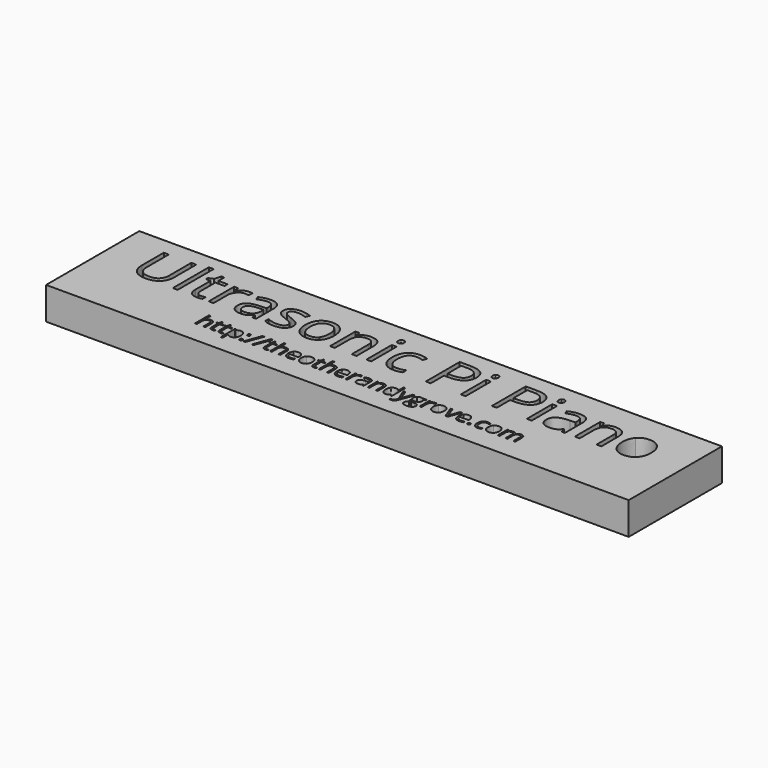
from build123d import *

# Parameters (mm, degrees)
F0_W     = 457.2
F0_H     = 91.44
F0_W_2   = 3.7731949911
F0_H_2   = 35.3546189624
F0_H_3   = 24.9001788909
F1_DEPTH = 25.4


with BuildPart() as f1:
    # F0 (on Top) → F1 (new body)
    with BuildSketch(Plane.XY):
        with Locations((-228.6, -172.72)):
            Rectangle(F0_W, F0_H)
        with BuildLine():
            add(Edge.make_bspline(
                [(-319.3360922734, -201.326012759), (-319.6287803103, -201.0501297769), (-319.6287803103, -200.4199402238)],
                knots=[0, 0, 0, 1, 1, 1], degree=2))
            add(Edge.make_bspline(
                [(-319.6287803103, -200.4199402238), (-319.6287803103, -199.8317633076), (-319.3612998555, -199.5306727434)],
                knots=[0, 0, 0, 1, 1, 1], degree=2))
            add(Edge.make_bspline(
                [(-319.3612998555, -199.5306727434), (-319.0938194008, -199.2295821791), (-318.5952694433, -199.2295821791)],
                knots=[0, 0, 0, 1, 1, 1], degree=2))
            add(Edge.make_bspline(
                [(-318.5952694433, -199.2295821791), (-318.0883169583, -199.2295821791), (-317.8040314488, -199.5306727434)],
                knots=[0, 0, 0, 1, 1, 1], degree=2))
            add(Edge.make_bspline(
                [(-317.8040314488, -199.5306727434), (-317.5197459393, -199.8317633076), (-317.5197459393, -200.4199402238)],
                knots=[0, 0, 0, 1, 1, 1], degree=2))
            add(Edge.make_bspline(
                [(-317.5197459393, -200.4199402238), (-317.5197459393, -200.9885112428), (-317.8082327125, -201.295203492)],
                knots=[0, 0, 0, 1, 1, 1], degree=2))
            add(Edge.make_bspline(
                [(-317.8082327125, -201.295203492), (-318.0967194857, -201.6018957411), (-318.5952694433, -201.6018957411)],
                knots=[0, 0, 0, 1, 1, 1], degree=2))
            add(Edge.make_bspline(
                [(-318.5952694433, -201.6018957411), (-319.0434042366, -201.6018957411), (-319.3360922734, -201.326012759)],
                knots=[0, 0, 0, 1, 1, 1], degree=2))
        make_face(mode=Mode.SUBTRACT)
        with BuildLine():
            add(Edge.make_bspline(
                [(-323.0107975785, -200.2140783031), (-324.065314764, -201.5234721523), (-325.9390783685, -201.5234721523)],
                knots=[0, 0, 0, 1, 1, 1], degree=2))
            add(Edge.make_bspline(
                [(-325.9390783685, -201.5234721523), (-326.8773605919, -201.5234721523), (-327.6517935316, -201.1775681087)],
                knots=[0, 0, 0, 1, 1, 1], degree=2))
            add(Edge.make_bspline(
                [(-327.6517935316, -201.1775681087), (-328.4262264713, -200.8316640652), (-328.9499840109, -200.1118475534)],
                knots=[0, 0, 0, 1, 1, 1], degree=2))
            Line((-328.9499840109, -200.1118475534), (-329.0564160243, -200.1118475534))
            add(Edge.make_bspline(
                [(-329.0564160243, -200.1118475534), (-328.9499840109, -200.9521002909), (-328.9499840109, -201.7055269121)],
                knots=[0, 0, 0, 1, 1, 1], degree=2))
            Line((-328.9499840109, -201.7055269121), (-328.9499840109, -205.654714778))
            Line((-328.9499840109, -205.654714778), (-330.4036212467, -205.654714778))
            Line((-330.4036212467, -205.654714778), (-330.4036212467, -191.7541336584))
            Line((-330.4036212467, -191.7541336584), (-329.2216657294, -191.7541336584))
            Line((-329.2216657294, -191.7541336584), (-329.0200050724, -193.0677287712))
            Line((-329.0200050724, -193.0677287712), (-328.9499840109, -193.0677287712))
            add(Edge.make_bspline(
                [(-328.9499840109, -193.0677287712), (-328.3898155193, -192.277891198), (-327.6461918467, -191.9277858908)],
                knots=[0, 0, 0, 1, 1, 1], degree=2))
            add(Edge.make_bspline(
                [(-327.6461918467, -191.9277858908), (-326.902568174, -191.5776805835), (-325.9390783685, -191.5776805835)],
                knots=[0, 0, 0, 1, 1, 1], degree=2))
            add(Edge.make_bspline(
                [(-325.9390783685, -191.5776805835), (-324.0317046545, -191.5776805835), (-322.9939925237, -192.882873169)],
                knots=[0, 0, 0, 1, 1, 1], degree=2))
            add(Edge.make_bspline(
                [(-322.9939925237, -192.882873169), (-321.956280393, -194.1880657545), (-321.956280393, -196.5407734193)],
                knots=[0, 0, 0, 1, 1, 1], degree=2))
            add(Edge.make_bspline(
                [(-321.956280393, -196.5407734193), (-321.956280393, -198.904684454), (-323.0107975785, -200.2140783031)],
                knots=[0, 0, 0, 1, 1, 1], degree=2))
        make_face(mode=Mode.SUBTRACT)
        with BuildLine():
            add(Edge.make_bspline(
                [(-278.445192806, -201.3778283445), (-279.1313992083, -201.5234721523), (-280.1032915412, -201.5234721523)],
                knots=[0, 0, 0, 1, 1, 1], degree=2))
            add(Edge.make_bspline(
                [(-280.1032915412, -201.5234721523), (-282.229130967, -201.5234721523), (-283.4601012273, -200.2266820942)],
                knots=[0, 0, 0, 1, 1, 1], degree=2))
            add(Edge.make_bspline(
                [(-283.4601012273, -200.2266820942), (-284.6910714876, -198.9298920361), (-284.6910714876, -196.630400378)],
                knots=[0, 0, 0, 1, 1, 1], degree=2))
            add(Edge.make_bspline(
                [(-284.6910714876, -196.630400378), (-284.6910714876, -194.3085019802), (-283.5483277647, -192.9430912818)],
                knots=[0, 0, 0, 1, 1, 1], degree=2))
            add(Edge.make_bspline(
                [(-283.5483277647, -192.9430912818), (-282.4055840418, -191.5776805835), (-280.4786044306, -191.5776805835)],
                knots=[0, 0, 0, 1, 1, 1], degree=2))
            add(Edge.make_bspline(
                [(-280.4786044306, -191.5776805835), (-278.67766273, -191.5776805835), (-277.6273468083, -192.7638373645)],
                knots=[0, 0, 0, 1, 1, 1], degree=2))
            add(Edge.make_bspline(
                [(-277.6273468083, -192.7638373645), (-276.5770308865, -193.9499941455), (-276.5770308865, -195.8937788115)],
                knots=[0, 0, 0, 1, 1, 1], degree=2))
            Line((-276.5770308865, -195.8937788115), (-276.5770308865, -196.8124551377))
            Line((-276.5770308865, -196.8124551377), (-283.1842182452, -196.8124551377))
            add(Edge.make_bspline(
                [(-283.1842182452, -196.8124551377), (-283.1394047658, -198.50136314), (-282.3299612954, -199.3766264082)],
                knots=[0, 0, 0, 1, 1, 1], degree=2))
            add(Edge.make_bspline(
                [(-282.3299612954, -199.3766264082), (-281.520517825, -200.2518896763), (-280.0500755345, -200.2518896763)],
                knots=[0, 0, 0, 1, 1, 1], degree=2))
            add(Edge.make_bspline(
                [(-280.0500755345, -200.2518896763), (-278.5012096552, -200.2518896763), (-276.9887547278, -199.6048950685)],
                knots=[0, 0, 0, 1, 1, 1], degree=2))
            Line((-276.9887547278, -199.6048950685), (-276.9887547278, -200.9016851266))
            add(Edge.make_bspline(
                [(-276.9887547278, -200.9016851266), (-277.7589864038, -201.2321845367), (-278.445192806, -201.3778283445)],
                knots=[0, 0, 0, 1, 1, 1], degree=2))
        make_face(mode=Mode.SUBTRACT)
        with BuildLine():
            add(Edge.make_bspline(
                [(-267.0051517858, -192.9178836997), (-265.8189950048, -194.2580868159), (-265.8189950048, -196.5407734193)],
                knots=[0, 0, 0, 1, 1, 1], degree=2))
            add(Edge.make_bspline(
                [(-265.8189950048, -196.5407734193), (-265.8189950048, -198.8878793992), (-266.9995501009, -200.2056757758)],
                knots=[0, 0, 0, 1, 1, 1], degree=2))
            add(Edge.make_bspline(
                [(-266.9995501009, -200.2056757758), (-268.180105197, -201.5234721523), (-270.2639319858, -201.5234721523)],
                knots=[0, 0, 0, 1, 1, 1], degree=2))
            add(Edge.make_bspline(
                [(-270.2639319858, -201.5234721523), (-271.5523195166, -201.5234721523), (-272.5494194317, -200.9184901814)],
                knots=[0, 0, 0, 1, 1, 1], degree=2))
            add(Edge.make_bspline(
                [(-272.5494194317, -200.9184901814), (-273.5465193468, -200.3135082104), (-274.0898827836, -199.1847686998)],
                knots=[0, 0, 0, 1, 1, 1], degree=2))
            add(Edge.make_bspline(
                [(-274.0898827836, -199.1847686998), (-274.6332462205, -198.0560291892), (-274.6332462205, -196.5407734193)],
                knots=[0, 0, 0, 1, 1, 1], degree=2))
            add(Edge.make_bspline(
                [(-274.6332462205, -196.5407734193), (-274.6332462205, -194.1964682819), (-273.4596932306, -192.8870744327)],
                knots=[0, 0, 0, 1, 1, 1], degree=2))
            add(Edge.make_bspline(
                [(-273.4596932306, -192.8870744327), (-272.2861402406, -191.5776805835), (-270.2023134518, -191.5776805835)],
                knots=[0, 0, 0, 1, 1, 1], degree=2))
            add(Edge.make_bspline(
                [(-270.2023134518, -191.5776805835), (-268.1913085668, -191.5776805835), (-267.0051517858, -192.9178836997)],
                knots=[0, 0, 0, 1, 1, 1], degree=2))
        make_face(mode=Mode.SUBTRACT)
        with BuildLine():
            add(Edge.make_bspline(
                [(-240.2304983074, -201.3778283445), (-240.9167047096, -201.5234721523), (-241.8885970426, -201.5234721523)],
                knots=[0, 0, 0, 1, 1, 1], degree=2))
            add(Edge.make_bspline(
                [(-241.8885970426, -201.5234721523), (-244.0144364683, -201.5234721523), (-245.2454067286, -200.2266820942)],
                knots=[0, 0, 0, 1, 1, 1], degree=2))
            add(Edge.make_bspline(
                [(-245.2454067286, -200.2266820942), (-246.476376989, -198.9298920361), (-246.476376989, -196.630400378)],
                knots=[0, 0, 0, 1, 1, 1], degree=2))
            add(Edge.make_bspline(
                [(-246.476376989, -196.630400378), (-246.476376989, -194.3085019802), (-245.3336332661, -192.9430912818)],
                knots=[0, 0, 0, 1, 1, 1], degree=2))
            add(Edge.make_bspline(
                [(-245.3336332661, -192.9430912818), (-244.1908895432, -191.5776805835), (-242.263909932, -191.5776805835)],
                knots=[0, 0, 0, 1, 1, 1], degree=2))
            add(Edge.make_bspline(
                [(-242.263909932, -191.5776805835), (-240.4629682314, -191.5776805835), (-239.4126523096, -192.7638373645)],
                knots=[0, 0, 0, 1, 1, 1], degree=2))
            add(Edge.make_bspline(
                [(-239.4126523096, -192.7638373645), (-238.3623363878, -193.9499941455), (-238.3623363878, -195.8937788115)],
                knots=[0, 0, 0, 1, 1, 1], degree=2))
            Line((-238.3623363878, -195.8937788115), (-238.3623363878, -196.8124551377))
            Line((-238.3623363878, -196.8124551377), (-244.9695237465, -196.8124551377))
            add(Edge.make_bspline(
                [(-244.9695237465, -196.8124551377), (-244.9247102672, -198.50136314), (-244.1152667968, -199.3766264082)],
                knots=[0, 0, 0, 1, 1, 1], degree=2))
            add(Edge.make_bspline(
                [(-244.1152667968, -199.3766264082), (-243.3058233264, -200.2518896763), (-241.8353810359, -200.2518896763)],
                knots=[0, 0, 0, 1, 1, 1], degree=2))
            add(Edge.make_bspline(
                [(-241.8353810359, -200.2518896763), (-240.2865151565, -200.2518896763), (-238.7740602291, -199.6048950685)],
                knots=[0, 0, 0, 1, 1, 1], degree=2))
            Line((-238.7740602291, -199.6048950685), (-238.7740602291, -200.9016851266))
            add(Edge.make_bspline(
                [(-238.7740602291, -200.9016851266), (-239.5442919051, -201.2321845367), (-240.2304983074, -201.3778283445)],
                knots=[0, 0, 0, 1, 1, 1], degree=2))
        make_face(mode=Mode.SUBTRACT)
        with BuildLine():
            add(Edge.make_bspline(
                [(-233.1611719431, -192.0860334897), (-232.4077453218, -191.5776805835), (-231.5058740503, -191.5776805835)],
                knots=[0, 0, 0, 1, 1, 1], degree=2))
            add(Edge.make_bspline(
                [(-231.5058740503, -191.5776805835), (-230.8672819699, -191.5776805835), (-230.3603294849, -191.6841125969)],
                knots=[0, 0, 0, 1, 1, 1], degree=2))
            Line((-230.3603294849, -191.6841125969), (-230.5619901419, -193.0313178193))
            add(Edge.make_bspline(
                [(-230.5619901419, -193.0313178193), (-231.155768743, -192.8996782237), (-231.6123060637, -192.8996782237)],
                knots=[0, 0, 0, 1, 1, 1], degree=2))
            add(Edge.make_bspline(
                [(-231.6123060637, -192.8996782237), (-232.7774565263, -192.8996782237), (-233.6037050514, -193.8449625534)],
                knots=[0, 0, 0, 1, 1, 1], degree=2))
            add(Edge.make_bspline(
                [(-233.6037050514, -193.8449625534), (-234.4299535766, -194.790246883), (-234.4299535766, -196.1990706394)],
                knots=[0, 0, 0, 1, 1, 1], degree=2))
            Line((-234.4299535766, -196.1990706394), (-234.4299535766, -201.3470190775))
            Line((-234.4299535766, -201.3470190775), (-235.8835908124, -201.3470190775))
            Line((-235.8835908124, -201.3470190775), (-235.8835908124, -191.7541336584))
            Line((-235.8835908124, -191.7541336584), (-234.6848302403, -191.7541336584))
            Line((-234.6848302403, -191.7541336584), (-234.5167796928, -193.5298677768))
            Line((-234.5167796928, -193.5298677768), (-234.4467586313, -193.5298677768))
            add(Edge.make_bspline(
                [(-234.4467586313, -193.5298677768), (-233.9145985643, -192.5943863958), (-233.1611719431, -192.0860334897)],
                knots=[0, 0, 0, 1, 1, 1], degree=2))
        make_face(mode=Mode.SUBTRACT)
        with BuildLine():
            Line((-346.0407246904, -201.3470190775), (-347.4943619262, -201.3470190775))
            Line((-347.4943619262, -201.3470190775), (-347.4943619262, -195.1403521902))
            add(Edge.make_bspline(
                [(-347.4943619262, -195.1403521902), (-347.4943619262, -193.9696000428), (-348.0279224145, -193.3912260751)],
                knots=[0, 0, 0, 1, 1, 1], degree=2))
            add(Edge.make_bspline(
                [(-348.0279224145, -193.3912260751), (-348.5614829027, -192.8128521075), (-349.7014257832, -192.8128521075)],
                knots=[0, 0, 0, 1, 1, 1], degree=2))
            add(Edge.make_bspline(
                [(-349.7014257832, -192.8128521075), (-351.2138807106, -192.8128521075), (-351.9098900614, -193.6362997902)],
                knots=[0, 0, 0, 1, 1, 1], degree=2))
            add(Edge.make_bspline(
                [(-351.9098900614, -193.6362997902), (-352.6058994123, -194.4597474729), (-352.6058994123, -196.330710235)],
                knots=[0, 0, 0, 1, 1, 1], degree=2))
            Line((-352.6058994123, -196.330710235), (-352.6058994123, -201.3470190775))
            Line((-352.6058994123, -201.3470190775), (-354.059536648, -201.3470190775))
            Line((-354.059536648, -201.3470190775), (-354.059536648, -187.7265222036))
            Line((-354.059536648, -187.7265222036), (-352.6058994123, -187.7265222036))
            Line((-352.6058994123, -187.7265222036), (-352.6058994123, -191.8493623019))
            add(Edge.make_bspline(
                [(-352.6058994123, -191.8493623019), (-352.6058994123, -192.5943863958), (-352.6759204737, -193.084533826)],
                knots=[0, 0, 0, 1, 1, 1], degree=2))
            Line((-352.6759204737, -193.084533826), (-352.5890943575, -193.084533826))
            add(Edge.make_bspline(
                [(-352.5890943575, -193.084533826), (-352.1605654614, -192.3927257388), (-351.3679270458, -191.9950061098)],
                knots=[0, 0, 0, 1, 1, 1], degree=2))
            add(Edge.make_bspline(
                [(-351.3679270458, -191.9950061098), (-350.5752886301, -191.5972864807), (-349.5613836603, -191.5972864807)],
                knots=[0, 0, 0, 1, 1, 1], degree=2))
            add(Edge.make_bspline(
                [(-349.5613836603, -191.5972864807), (-347.8024545966, -191.5972864807), (-346.9215896435, -192.4333379545)],
                knots=[0, 0, 0, 1, 1, 1], degree=2))
            add(Edge.make_bspline(
                [(-346.9215896435, -192.4333379545), (-346.0407246904, -193.2693894282), (-346.0407246904, -195.089937026)],
                knots=[0, 0, 0, 1, 1, 1], degree=2))
            Line((-346.0407246904, -195.089937026), (-346.0407246904, -201.3470190775))
        make_face(mode=Mode.SUBTRACT)
        with BuildLine():
            add(Edge.make_bspline(
                [(-341.0888352245, -199.858371311), (-340.6771113831, -200.3219107378), (-339.9600957138, -200.3219107378)],
                knots=[0, 0, 0, 1, 1, 1], degree=2))
            add(Edge.make_bspline(
                [(-339.9600957138, -200.3219107378), (-339.5735794546, -200.3219107378), (-339.21507162, -200.2658938886)],
                knots=[0, 0, 0, 1, 1, 1], degree=2))
            add(Edge.make_bspline(
                [(-339.21507162, -200.2658938886), (-338.8565637853, -200.2098770395), (-338.646500601, -200.1482585054)],
                knots=[0, 0, 0, 1, 1, 1], degree=2))
            Line((-338.646500601, -200.1482585054), (-338.646500601, -201.2601929613))
            add(Edge.make_bspline(
                [(-338.646500601, -201.2601929613), (-338.8817713675, -201.3722266596), (-339.3411095306, -201.4478494059)],
                knots=[0, 0, 0, 1, 1, 1], degree=2))
            add(Edge.make_bspline(
                [(-339.3411095306, -201.4478494059), (-339.8004476937, -201.5234721523), (-340.1701588982, -201.5234721523)],
                knots=[0, 0, 0, 1, 1, 1], degree=2))
            add(Edge.make_bspline(
                [(-340.1701588982, -201.5234721523), (-342.9513954591, -201.5234721523), (-342.9513954591, -198.5909900987)],
                knots=[0, 0, 0, 1, 1, 1], degree=2))
            Line((-342.9513954591, -198.5909900987), (-342.9513954591, -192.882873169))
            Line((-342.9513954591, -192.882873169), (-344.326609106, -192.882873169))
            Line((-344.326609106, -192.882873169), (-344.326609106, -192.1826625545))
            Line((-344.326609106, -192.1826625545), (-342.9513954591, -191.5776805835))
            Line((-342.9513954591, -191.5776805835), (-342.3408118032, -189.5302647466))
            Line((-342.3408118032, -189.5302647466), (-341.5005590658, -189.5302647466))
            Line((-341.5005590658, -189.5302647466), (-341.5005590658, -191.7541336584))
            Line((-341.5005590658, -191.7541336584), (-338.7165216624, -191.7541336584))
            Line((-338.7165216624, -191.7541336584), (-338.7165216624, -192.882873169))
            Line((-338.7165216624, -192.882873169), (-341.5005590658, -192.882873169))
            Line((-341.5005590658, -192.882873169), (-341.5005590658, -198.5293715646))
            add(Edge.make_bspline(
                [(-341.5005590658, -198.5293715646), (-341.5005590658, -199.3948318841), (-341.0888352245, -199.858371311)],
                knots=[0, 0, 0, 1, 1, 1], degree=2))
        make_face(mode=Mode.SUBTRACT)
        with BuildLine():
            add(Edge.make_bspline(
                [(-334.7617321115, -199.858371311), (-334.3500082702, -200.3219107378), (-333.6329926009, -200.3219107378)],
                knots=[0, 0, 0, 1, 1, 1], degree=2))
            add(Edge.make_bspline(
                [(-333.6329926009, -200.3219107378), (-333.2464763417, -200.3219107378), (-332.8879685071, -200.2658938886)],
                knots=[0, 0, 0, 1, 1, 1], degree=2))
            add(Edge.make_bspline(
                [(-332.8879685071, -200.2658938886), (-332.5294606724, -200.2098770395), (-332.3193974881, -200.1482585054)],
                knots=[0, 0, 0, 1, 1, 1], degree=2))
            Line((-332.3193974881, -200.1482585054), (-332.3193974881, -201.2601929613))
            add(Edge.make_bspline(
                [(-332.3193974881, -201.2601929613), (-332.5546682545, -201.3722266596), (-333.0140064177, -201.4478494059)],
                knots=[0, 0, 0, 1, 1, 1], degree=2))
            add(Edge.make_bspline(
                [(-333.0140064177, -201.4478494059), (-333.4733445808, -201.5234721523), (-333.8430557853, -201.5234721523)],
                knots=[0, 0, 0, 1, 1, 1], degree=2))
            add(Edge.make_bspline(
                [(-333.8430557853, -201.5234721523), (-336.6242923462, -201.5234721523), (-336.6242923462, -198.5909900987)],
                knots=[0, 0, 0, 1, 1, 1], degree=2))
            Line((-336.6242923462, -198.5909900987), (-336.6242923462, -192.882873169))
            Line((-336.6242923462, -192.882873169), (-337.9995059931, -192.882873169))
            Line((-337.9995059931, -192.882873169), (-337.9995059931, -192.1826625545))
            Line((-337.9995059931, -192.1826625545), (-336.6242923462, -191.5776805835))
            Line((-336.6242923462, -191.5776805835), (-336.0137086903, -189.5302647466))
            Line((-336.0137086903, -189.5302647466), (-335.1734559529, -189.5302647466))
            Line((-335.1734559529, -189.5302647466), (-335.1734559529, -191.7541336584))
            Line((-335.1734559529, -191.7541336584), (-332.3894185495, -191.7541336584))
            Line((-332.3894185495, -191.7541336584), (-332.3894185495, -192.882873169))
            Line((-332.3894185495, -192.882873169), (-335.1734559529, -192.882873169))
            Line((-335.1734559529, -192.882873169), (-335.1734559529, -198.5293715646))
            add(Edge.make_bspline(
                [(-335.1734559529, -198.5293715646), (-335.1734559529, -199.3948318841), (-334.7617321115, -199.858371311)],
                knots=[0, 0, 0, 1, 1, 1], degree=2))
        make_face(mode=Mode.SUBTRACT)
        with BuildLine():
            add(Edge.make_bspline(
                [(-319.3360922734, -193.5956875746), (-319.6287803103, -193.3198045925), (-319.6287803103, -192.6896150394)],
                knots=[0, 0, 0, 1, 1, 1], degree=2))
            add(Edge.make_bspline(
                [(-319.6287803103, -192.6896150394), (-319.6287803103, -191.5076595221), (-318.5952694433, -191.5076595221)],
                knots=[0, 0, 0, 1, 1, 1], degree=2))
            add(Edge.make_bspline(
                [(-318.5952694433, -191.5076595221), (-317.5197459393, -191.5076595221), (-317.5197459393, -192.6896150394)],
                knots=[0, 0, 0, 1, 1, 1], degree=2))
            add(Edge.make_bspline(
                [(-317.5197459393, -192.6896150394), (-317.5197459393, -193.2581860584), (-317.8082327125, -193.5648783076)],
                knots=[0, 0, 0, 1, 1, 1], degree=2))
            add(Edge.make_bspline(
                [(-317.8082327125, -193.5648783076), (-318.0967194857, -193.8715705567), (-318.5952694433, -193.8715705567)],
                knots=[0, 0, 0, 1, 1, 1], degree=2))
            add(Edge.make_bspline(
                [(-318.5952694433, -193.8715705567), (-319.0434042366, -193.8715705567), (-319.3360922734, -193.5956875746)],
                knots=[0, 0, 0, 1, 1, 1], degree=2))
        make_face(mode=Mode.SUBTRACT)
        Polygon((-311.2430579907, -188.5499698863), (-309.7922215974, -188.5499698863), (-314.5620563035, -201.3470190775), (-316.0128926969, -201.3470190775), align=None, mode=Mode.SUBTRACT)
        Polygon((-304.6610782141, -188.5499698863), (-303.2102418208, -188.5499698863), (-307.980076527, -201.3470190775), (-309.4309129203, -201.3470190775), align=None, mode=Mode.SUBTRACT)
        with BuildLine():
            add(Edge.make_bspline(
                [(-299.5159306185, -199.858371311), (-299.1042067772, -200.3219107378), (-298.3871911079, -200.3219107378)],
                knots=[0, 0, 0, 1, 1, 1], degree=2))
            add(Edge.make_bspline(
                [(-298.3871911079, -200.3219107378), (-298.0006748487, -200.3219107378), (-297.642167014, -200.2658938886)],
                knots=[0, 0, 0, 1, 1, 1], degree=2))
            add(Edge.make_bspline(
                [(-297.642167014, -200.2658938886), (-297.2836591794, -200.2098770395), (-297.073595995, -200.1482585054)],
                knots=[0, 0, 0, 1, 1, 1], degree=2))
            Line((-297.073595995, -200.1482585054), (-297.073595995, -201.2601929613))
            add(Edge.make_bspline(
                [(-297.073595995, -201.2601929613), (-297.3088667615, -201.3722266596), (-297.7682049246, -201.4478494059)],
                knots=[0, 0, 0, 1, 1, 1], degree=2))
            add(Edge.make_bspline(
                [(-297.7682049246, -201.4478494059), (-298.2275430878, -201.5234721523), (-298.5972542922, -201.5234721523)],
                knots=[0, 0, 0, 1, 1, 1], degree=2))
            add(Edge.make_bspline(
                [(-298.5972542922, -201.5234721523), (-301.3784908532, -201.5234721523), (-301.3784908532, -198.5909900987)],
                knots=[0, 0, 0, 1, 1, 1], degree=2))
            Line((-301.3784908532, -198.5909900987), (-301.3784908532, -192.882873169))
            Line((-301.3784908532, -192.882873169), (-302.7537045001, -192.882873169))
            Line((-302.7537045001, -192.882873169), (-302.7537045001, -192.1826625545))
            Line((-302.7537045001, -192.1826625545), (-301.3784908532, -191.5776805835))
            Line((-301.3784908532, -191.5776805835), (-300.7679071973, -189.5302647466))
            Line((-300.7679071973, -189.5302647466), (-299.9276544598, -189.5302647466))
            Line((-299.9276544598, -189.5302647466), (-299.9276544598, -191.7541336584))
            Line((-299.9276544598, -191.7541336584), (-297.1436170565, -191.7541336584))
            Line((-297.1436170565, -191.7541336584), (-297.1436170565, -192.882873169))
            Line((-297.1436170565, -192.882873169), (-299.9276544598, -192.882873169))
            Line((-299.9276544598, -192.882873169), (-299.9276544598, -198.5293715646))
            add(Edge.make_bspline(
                [(-299.9276544598, -198.5293715646), (-299.9276544598, -199.3948318841), (-299.5159306185, -199.858371311)],
                knots=[0, 0, 0, 1, 1, 1], degree=2))
        make_face(mode=Mode.SUBTRACT)
        with BuildLine():
            Line((-287.139007796, -201.3470190775), (-288.5926450318, -201.3470190775))
            Line((-288.5926450318, -201.3470190775), (-288.5926450318, -195.1403521902))
            add(Edge.make_bspline(
                [(-288.5926450318, -195.1403521902), (-288.5926450318, -193.9696000428), (-289.1262055201, -193.3912260751)],
                knots=[0, 0, 0, 1, 1, 1], degree=2))
            add(Edge.make_bspline(
                [(-289.1262055201, -193.3912260751), (-289.6597660084, -192.8128521075), (-290.7997088888, -192.8128521075)],
                knots=[0, 0, 0, 1, 1, 1], degree=2))
            add(Edge.make_bspline(
                [(-290.7997088888, -192.8128521075), (-292.3121638162, -192.8128521075), (-293.008173167, -193.6362997902)],
                knots=[0, 0, 0, 1, 1, 1], degree=2))
            add(Edge.make_bspline(
                [(-293.008173167, -193.6362997902), (-293.7041825179, -194.4597474729), (-293.7041825179, -196.330710235)],
                knots=[0, 0, 0, 1, 1, 1], degree=2))
            Line((-293.7041825179, -196.330710235), (-293.7041825179, -201.3470190775))
            Line((-293.7041825179, -201.3470190775), (-295.1578197537, -201.3470190775))
            Line((-295.1578197537, -201.3470190775), (-295.1578197537, -187.7265222036))
            Line((-295.1578197537, -187.7265222036), (-293.7041825179, -187.7265222036))
            Line((-293.7041825179, -187.7265222036), (-293.7041825179, -191.8493623019))
            add(Edge.make_bspline(
                [(-293.7041825179, -191.8493623019), (-293.7041825179, -192.5943863958), (-293.7742035793, -193.084533826)],
                knots=[0, 0, 0, 1, 1, 1], degree=2))
            Line((-293.7742035793, -193.084533826), (-293.6873774631, -193.084533826))
            add(Edge.make_bspline(
                [(-293.6873774631, -193.084533826), (-293.258848567, -192.3927257388), (-292.4662101514, -191.9950061098)],
                knots=[0, 0, 0, 1, 1, 1], degree=2))
            add(Edge.make_bspline(
                [(-292.4662101514, -191.9950061098), (-291.6735717358, -191.5972864807), (-290.6596667659, -191.5972864807)],
                knots=[0, 0, 0, 1, 1, 1], degree=2))
            add(Edge.make_bspline(
                [(-290.6596667659, -191.5972864807), (-288.9007377022, -191.5972864807), (-288.0198727491, -192.4333379545)],
                knots=[0, 0, 0, 1, 1, 1], degree=2))
            add(Edge.make_bspline(
                [(-288.0198727491, -192.4333379545), (-287.139007796, -193.2693894282), (-287.139007796, -195.089937026)],
                knots=[0, 0, 0, 1, 1, 1], degree=2))
            Line((-287.139007796, -195.089937026), (-287.139007796, -201.3470190775))
        make_face(mode=Mode.SUBTRACT)
        with BuildLine():
            add(Edge.make_bspline(
                [(-261.3012361198, -199.858371311), (-260.8895122785, -200.3219107378), (-260.1724966092, -200.3219107378)],
                knots=[0, 0, 0, 1, 1, 1], degree=2))
            add(Edge.make_bspline(
                [(-260.1724966092, -200.3219107378), (-259.78598035, -200.3219107378), (-259.4274725154, -200.2658938886)],
                knots=[0, 0, 0, 1, 1, 1], degree=2))
            add(Edge.make_bspline(
                [(-259.4274725154, -200.2658938886), (-259.0689646807, -200.2098770395), (-258.8589014964, -200.1482585054)],
                knots=[0, 0, 0, 1, 1, 1], degree=2))
            Line((-258.8589014964, -200.1482585054), (-258.8589014964, -201.2601929613))
            add(Edge.make_bspline(
                [(-258.8589014964, -201.2601929613), (-259.0941722628, -201.3722266596), (-259.553510426, -201.4478494059)],
                knots=[0, 0, 0, 1, 1, 1], degree=2))
            add(Edge.make_bspline(
                [(-259.553510426, -201.4478494059), (-260.0128485891, -201.5234721523), (-260.3825597936, -201.5234721523)],
                knots=[0, 0, 0, 1, 1, 1], degree=2))
            add(Edge.make_bspline(
                [(-260.3825597936, -201.5234721523), (-263.1637963545, -201.5234721523), (-263.1637963545, -198.5909900987)],
                knots=[0, 0, 0, 1, 1, 1], degree=2))
            Line((-263.1637963545, -198.5909900987), (-263.1637963545, -192.882873169))
            Line((-263.1637963545, -192.882873169), (-264.5390100014, -192.882873169))
            Line((-264.5390100014, -192.882873169), (-264.5390100014, -192.1826625545))
            Line((-264.5390100014, -192.1826625545), (-263.1637963545, -191.5776805835))
            Line((-263.1637963545, -191.5776805835), (-262.5532126986, -189.5302647466))
            Line((-262.5532126986, -189.5302647466), (-261.7129599612, -189.5302647466))
            Line((-261.7129599612, -189.5302647466), (-261.7129599612, -191.7541336584))
            Line((-261.7129599612, -191.7541336584), (-258.9289225578, -191.7541336584))
            Line((-258.9289225578, -191.7541336584), (-258.9289225578, -192.882873169))
            Line((-258.9289225578, -192.882873169), (-261.7129599612, -192.882873169))
            Line((-261.7129599612, -192.882873169), (-261.7129599612, -198.5293715646))
            add(Edge.make_bspline(
                [(-261.7129599612, -198.5293715646), (-261.7129599612, -199.3948318841), (-261.3012361198, -199.858371311)],
                knots=[0, 0, 0, 1, 1, 1], degree=2))
        make_face(mode=Mode.SUBTRACT)
        with BuildLine():
            Line((-248.9243132974, -201.3470190775), (-250.3779505332, -201.3470190775))
            Line((-250.3779505332, -201.3470190775), (-250.3779505332, -195.1403521902))
            add(Edge.make_bspline(
                [(-250.3779505332, -195.1403521902), (-250.3779505332, -193.9696000428), (-250.9115110214, -193.3912260751)],
                knots=[0, 0, 0, 1, 1, 1], degree=2))
            add(Edge.make_bspline(
                [(-250.9115110214, -193.3912260751), (-251.4450715097, -192.8128521075), (-252.5850143902, -192.8128521075)],
                knots=[0, 0, 0, 1, 1, 1], degree=2))
            add(Edge.make_bspline(
                [(-252.5850143902, -192.8128521075), (-254.0974693175, -192.8128521075), (-254.7934786684, -193.6362997902)],
                knots=[0, 0, 0, 1, 1, 1], degree=2))
            add(Edge.make_bspline(
                [(-254.7934786684, -193.6362997902), (-255.4894880192, -194.4597474729), (-255.4894880192, -196.330710235)],
                knots=[0, 0, 0, 1, 1, 1], degree=2))
            Line((-255.4894880192, -196.330710235), (-255.4894880192, -201.3470190775))
            Line((-255.4894880192, -201.3470190775), (-256.943125255, -201.3470190775))
            Line((-256.943125255, -201.3470190775), (-256.943125255, -187.7265222036))
            Line((-256.943125255, -187.7265222036), (-255.4894880192, -187.7265222036))
            Line((-255.4894880192, -187.7265222036), (-255.4894880192, -191.8493623019))
            add(Edge.make_bspline(
                [(-255.4894880192, -191.8493623019), (-255.4894880192, -192.5943863958), (-255.5595090807, -193.084533826)],
                knots=[0, 0, 0, 1, 1, 1], degree=2))
            Line((-255.5595090807, -193.084533826), (-255.4726829645, -193.084533826))
            add(Edge.make_bspline(
                [(-255.4726829645, -193.084533826), (-255.0441540684, -192.3927257388), (-254.2515156527, -191.9950061098)],
                knots=[0, 0, 0, 1, 1, 1], degree=2))
            add(Edge.make_bspline(
                [(-254.2515156527, -191.9950061098), (-253.4588772371, -191.5972864807), (-252.4449722672, -191.5972864807)],
                knots=[0, 0, 0, 1, 1, 1], degree=2))
            add(Edge.make_bspline(
                [(-252.4449722672, -191.5972864807), (-250.6860432035, -191.5972864807), (-249.8051782505, -192.4333379545)],
                knots=[0, 0, 0, 1, 1, 1], degree=2))
            add(Edge.make_bspline(
                [(-249.8051782505, -192.4333379545), (-248.9243132974, -193.2693894282), (-248.9243132974, -195.089937026)],
                knots=[0, 0, 0, 1, 1, 1], degree=2))
            Line((-248.9243132974, -195.089937026), (-248.9243132974, -201.3470190775))
        make_face(mode=Mode.SUBTRACT)
        with BuildLine():
            Line((-221.5880909061, -201.3470190775), (-222.6664152525, -201.3470190775))
            Line((-222.6664152525, -201.3470190775), (-222.9549020256, -199.9802079579))
            Line((-222.9549020256, -199.9802079579), (-223.0249230871, -199.9802079579))
            add(Edge.make_bspline(
                [(-223.0249230871, -199.9802079579), (-223.7419387564, -200.8820792294), (-224.454753162, -201.2027756909)],
                knots=[0, 0, 0, 1, 1, 1], degree=2))
            add(Edge.make_bspline(
                [(-224.454753162, -201.2027756909), (-225.1675675676, -201.5234721523), (-226.2374893866, -201.5234721523)],
                knots=[0, 0, 0, 1, 1, 1], degree=2))
            add(Edge.make_bspline(
                [(-226.2374893866, -201.5234721523), (-227.6631181978, -201.5234721523), (-228.4725616682, -200.7868505858)],
                knots=[0, 0, 0, 1, 1, 1], degree=2))
            add(Edge.make_bspline(
                [(-228.4725616682, -200.7868505858), (-229.2820051386, -200.0502290193), (-229.2820051386, -198.6946212696)],
                knots=[0, 0, 0, 1, 1, 1], degree=2))
            add(Edge.make_bspline(
                [(-229.2820051386, -198.6946212696), (-229.2820051386, -195.7901476405), (-224.6354075005, -195.6501055176)],
                knots=[0, 0, 0, 1, 1, 1], degree=2))
            Line((-224.6354075005, -195.6501055176), (-223.0081180324, -195.5968895109))
            Line((-223.0081180324, -195.5968895109), (-223.0081180324, -195.0003100673))
            add(Edge.make_bspline(
                [(-223.0081180324, -195.0003100673), (-223.0081180324, -193.8715705567), (-223.4926637776, -193.3338088048)],
                knots=[0, 0, 0, 1, 1, 1], degree=2))
            add(Edge.make_bspline(
                [(-223.4926637776, -193.3338088048), (-223.9772095229, -192.7960470528), (-225.0471313419, -192.7960470528)],
                knots=[0, 0, 0, 1, 1, 1], degree=2))
            add(Edge.make_bspline(
                [(-225.0471313419, -192.7960470528), (-226.2458919139, -192.7960470528), (-227.7583468413, -193.5298677768)],
                knots=[0, 0, 0, 1, 1, 1], degree=2))
            Line((-227.7583468413, -193.5298677768), (-228.2064816346, -192.4179333209))
            add(Edge.make_bspline(
                [(-228.2064816346, -192.4179333209), (-227.4978684927, -192.0342179042), (-226.6534144916, -191.8157521925)],
                knots=[0, 0, 0, 1, 1, 1], degree=2))
            add(Edge.make_bspline(
                [(-226.6534144916, -191.8157521925), (-225.8089604905, -191.5972864807), (-224.9575043832, -191.5972864807)],
                knots=[0, 0, 0, 1, 1, 1], degree=2))
            add(Edge.make_bspline(
                [(-224.9575043832, -191.5972864807), (-223.2433887988, -191.5972864807), (-222.4157398525, -192.3577152081)],
                knots=[0, 0, 0, 1, 1, 1], degree=2))
            add(Edge.make_bspline(
                [(-222.4157398525, -192.3577152081), (-221.5880909061, -193.1181439355), (-221.5880909061, -194.7986494104)],
                knots=[0, 0, 0, 1, 1, 1], degree=2))
            Line((-221.5880909061, -194.7986494104), (-221.5880909061, -201.3470190775))
        make_face(mode=Mode.SUBTRACT)
        with BuildLine():
            Line((-210.5779792032, -201.3470190775), (-212.031616439, -201.3470190775))
            Line((-212.031616439, -201.3470190775), (-212.031616439, -195.1403521902))
            add(Edge.make_bspline(
                [(-212.031616439, -195.1403521902), (-212.031616439, -193.9696000428), (-212.5651769272, -193.3912260751)],
                knots=[0, 0, 0, 1, 1, 1], degree=2))
            add(Edge.make_bspline(
                [(-212.5651769272, -193.3912260751), (-213.0987374155, -192.8128521075), (-214.238680296, -192.8128521075)],
                knots=[0, 0, 0, 1, 1, 1], degree=2))
            add(Edge.make_bspline(
                [(-214.238680296, -192.8128521075), (-215.742732696, -192.8128521075), (-216.4429433105, -193.6264968416)],
                knots=[0, 0, 0, 1, 1, 1], degree=2))
            add(Edge.make_bspline(
                [(-216.4429433105, -193.6264968416), (-217.143153925, -194.4401415757), (-217.143153925, -196.3139051802)],
                knots=[0, 0, 0, 1, 1, 1], degree=2))
            Line((-217.143153925, -196.3139051802), (-217.143153925, -201.3470190775))
            Line((-217.143153925, -201.3470190775), (-218.5967911608, -201.3470190775))
            Line((-218.5967911608, -201.3470190775), (-218.5967911608, -191.7541336584))
            Line((-218.5967911608, -191.7541336584), (-217.4148356435, -191.7541336584))
            Line((-217.4148356435, -191.7541336584), (-217.179564877, -193.0677287712))
            Line((-217.179564877, -193.0677287712), (-217.1095438155, -193.0677287712))
            add(Edge.make_bspline(
                [(-217.1095438155, -193.0677287712), (-216.6614090222, -192.3591156293), (-215.8561668155, -191.9683981064)],
                knots=[0, 0, 0, 1, 1, 1], degree=2))
            add(Edge.make_bspline(
                [(-215.8561668155, -191.9683981064), (-215.0509246088, -191.5776805835), (-214.0622272211, -191.5776805835)],
                knots=[0, 0, 0, 1, 1, 1], degree=2))
            add(Edge.make_bspline(
                [(-214.0622272211, -191.5776805835), (-212.3285057395, -191.5776805835), (-211.4532424714, -192.4137320573)],
                knots=[0, 0, 0, 1, 1, 1], degree=2))
            add(Edge.make_bspline(
                [(-211.4532424714, -192.4137320573), (-210.5779792032, -193.249783531), (-210.5779792032, -195.089937026)],
                knots=[0, 0, 0, 1, 1, 1], degree=2))
            Line((-210.5779792032, -195.089937026), (-210.5779792032, -201.3470190775))
        make_face(mode=Mode.SUBTRACT)
        with BuildLine():
            Line((-194.2630718846, -201.4002350842), (-198.1338361617, -191.7541336584))
            Line((-198.1338361617, -191.7541336584), (-196.5737669126, -191.7541336584))
            Line((-196.5737669126, -191.7541336584), (-194.473135069, -197.2241789791))
            add(Edge.make_bspline(
                [(-194.473135069, -197.2241789791), (-193.7841278243, -199.0979425836), (-193.6160772768, -199.9297927936)],
                knots=[0, 0, 0, 1, 1, 1], degree=2))
            Line((-193.6160772768, -199.9297927936), (-193.5460562153, -199.9297927936))
            add(Edge.make_bspline(
                [(-193.5460562153, -199.9297927936), (-193.434022517, -199.4816580003), (-193.0699129975, -198.4005328115)],
                knots=[0, 0, 0, 1, 1, 1], degree=2))
            add(Edge.make_bspline(
                [(-193.0699129975, -198.4005328115), (-192.7058034779, -197.3194076227), (-190.6919977505, -191.7541336584)],
                knots=[0, 0, 0, 1, 1, 1], degree=2))
            Line((-190.6919977505, -191.7541336584), (-189.1347293438, -191.7541336584))
            Line((-189.1347293438, -191.7541336584), (-193.2575694421, -202.6774192451))
            add(Edge.make_bspline(
                [(-193.2575694421, -202.6774192451), (-193.8709539405, -204.2963061859), (-194.6887999382, -204.975510482)],
                knots=[0, 0, 0, 1, 1, 1], degree=2))
            add(Edge.make_bspline(
                [(-194.6887999382, -204.975510482), (-195.506645936, -205.654714778), (-196.6970039807, -205.654714778)],
                knots=[0, 0, 0, 1, 1, 1], degree=2))
            add(Edge.make_bspline(
                [(-196.6970039807, -205.654714778), (-197.3636044858, -205.654714778), (-198.0105990936, -205.5034692853)],
                knots=[0, 0, 0, 1, 1, 1], degree=2))
            Line((-198.0105990936, -205.5034692853), (-198.0105990936, -204.3411196652))
            add(Edge.make_bspline(
                [(-198.0105990936, -204.3411196652), (-197.5288541908, -204.4447508361), (-196.9350755897, -204.4447508361)],
                knots=[0, 0, 0, 1, 1, 1], degree=2))
            add(Edge.make_bspline(
                [(-196.9350755897, -204.4447508361), (-195.4366248746, -204.4447508361), (-194.7980327941, -202.7642453613)],
                knots=[0, 0, 0, 1, 1, 1], degree=2))
            Line((-194.7980327941, -202.7642453613), (-194.2630718846, -201.4002350842))
        make_face(mode=Mode.SUBTRACT)
        with BuildLine():
            Line((-183.0428969974, -191.7541336584), (-179.7266995269, -191.7541336584))
            Line((-179.7266995269, -191.7541336584), (-179.7266995269, -192.6728099846))
            Line((-179.7266995269, -192.6728099846), (-181.5024336454, -192.882873169))
            add(Edge.make_bspline(
                [(-181.5024336454, -192.882873169), (-181.2587603515, -193.1881649969), (-181.0655022219, -193.683914112)],
                knots=[0, 0, 0, 1, 1, 1], degree=2))
            add(Edge.make_bspline(
                [(-181.0655022219, -193.683914112), (-180.8722440923, -194.1796632271), (-180.8722440923, -194.7986494104)],
                knots=[0, 0, 0, 1, 1, 1], degree=2))
            add(Edge.make_bspline(
                [(-180.8722440923, -194.7986494104), (-180.8722440923, -196.2102740093), (-181.8357338979, -197.0505267467)],
                knots=[0, 0, 0, 1, 1, 1], degree=2))
            add(Edge.make_bspline(
                [(-181.8357338979, -197.0505267467), (-182.7992237035, -197.8907794841), (-184.4797291784, -197.8907794841)],
                knots=[0, 0, 0, 1, 1, 1], degree=2))
            add(Edge.make_bspline(
                [(-184.4797291784, -197.8907794841), (-184.9082580745, -197.8907794841), (-185.2835709639, -197.8207584227)],
                knots=[0, 0, 0, 1, 1, 1], degree=2))
            add(Edge.make_bspline(
                [(-185.2835709639, -197.8207584227), (-186.2106498175, -198.3109058528), (-186.2106498175, -199.0531291042)],
                knots=[0, 0, 0, 1, 1, 1], degree=2))
            add(Edge.make_bspline(
                [(-186.2106498175, -199.0531291042), (-186.2106498175, -199.4480478908), (-185.8871525136, -199.6357043355)],
                knots=[0, 0, 0, 1, 1, 1], degree=2))
            add(Edge.make_bspline(
                [(-185.8871525136, -199.6357043355), (-185.5636552097, -199.8233607802), (-184.7766184789, -199.8233607802)],
                knots=[0, 0, 0, 1, 1, 1], degree=2))
            Line((-184.7766184789, -199.8233607802), (-183.0793079493, -199.8233607802))
            add(Edge.make_bspline(
                [(-183.0793079493, -199.8233607802), (-181.5192387001, -199.8233607802), (-180.6845876476, -200.4801583367)],
                knots=[0, 0, 0, 1, 1, 1], degree=2))
            add(Edge.make_bspline(
                [(-180.6845876476, -200.4801583367), (-179.8499365951, -201.1369558931), (-179.8499365951, -202.3889324719)],
                knots=[0, 0, 0, 1, 1, 1], degree=2))
            add(Edge.make_bspline(
                [(-179.8499365951, -202.3889324719), (-179.8499365951, -203.9826118305), (-181.127120756, -204.8186633043)],
                knots=[0, 0, 0, 1, 1, 1], degree=2))
            add(Edge.make_bspline(
                [(-181.127120756, -204.8186633043), (-182.4043049169, -205.654714778), (-184.8550420678, -205.654714778)],
                knots=[0, 0, 0, 1, 1, 1], degree=2))
            add(Edge.make_bspline(
                [(-184.8550420678, -205.654714778), (-186.7372081996, -205.654714778), (-187.7567148544, -204.9545041635)],
                knots=[0, 0, 0, 1, 1, 1], degree=2))
            add(Edge.make_bspline(
                [(-187.7567148544, -204.9545041635), (-188.7762215091, -204.254293549), (-188.7762215091, -202.9743085456)],
                knots=[0, 0, 0, 1, 1, 1], degree=2))
            add(Edge.make_bspline(
                [(-188.7762215091, -202.9743085456), (-188.7762215091, -202.1004456987), (-188.2160530175, -201.460453197)],
                knots=[0, 0, 0, 1, 1, 1], degree=2))
            add(Edge.make_bspline(
                [(-188.2160530175, -201.460453197), (-187.6558845259, -200.8204606953), (-186.6419795561, -200.5935924562)],
                knots=[0, 0, 0, 1, 1, 1], degree=2))
            add(Edge.make_bspline(
                [(-186.6419795561, -200.5935924562), (-187.0088899181, -200.4283427512), (-187.2581648968, -200.0782374439)],
                knots=[0, 0, 0, 1, 1, 1], degree=2))
            add(Edge.make_bspline(
                [(-187.2581648968, -200.0782374439), (-187.5074398756, -199.7281321367), (-187.5074398756, -199.2631922886)],
                knots=[0, 0, 0, 1, 1, 1], degree=2))
            add(Edge.make_bspline(
                [(-187.5074398756, -199.2631922886), (-187.5074398756, -198.7394347489), (-187.2273556298, -198.3445159623)],
                knots=[0, 0, 0, 1, 1, 1], degree=2))
            add(Edge.make_bspline(
                [(-187.2273556298, -198.3445159623), (-186.947271384, -197.9495971757), (-186.342289413, -197.5826868137)],
                knots=[0, 0, 0, 1, 1, 1], degree=2))
            add(Edge.make_bspline(
                [(-186.342289413, -197.5826868137), (-187.0873135069, -197.2773949858), (-187.5550541974, -196.5421738405)],
                knots=[0, 0, 0, 1, 1, 1], degree=2))
            add(Edge.make_bspline(
                [(-187.5550541974, -196.5421738405), (-188.0227948879, -195.8069526953), (-188.0227948879, -194.8602679444)],
                knots=[0, 0, 0, 1, 1, 1], degree=2))
            add(Edge.make_bspline(
                [(-188.0227948879, -194.8602679444), (-188.0227948879, -193.286194483), (-187.0775105583, -192.4319375332)],
                knots=[0, 0, 0, 1, 1, 1], degree=2))
            add(Edge.make_bspline(
                [(-187.0775105583, -192.4319375332), (-186.1322262287, -191.5776805835), (-184.4013055896, -191.5776805835)],
                knots=[0, 0, 0, 1, 1, 1], degree=2))
            add(Edge.make_bspline(
                [(-184.4013055896, -191.5776805835), (-183.6478789683, -191.5776805835), (-183.0428969974, -191.7541336584)],
                knots=[0, 0, 0, 1, 1, 1], degree=2))
        make_face(mode=Mode.SUBTRACT)
        with BuildLine():
            add(Edge.make_bspline(
                [(-175.0352884096, -192.0860334897), (-174.2818617883, -191.5776805835), (-173.3799905168, -191.5776805835)],
                knots=[0, 0, 0, 1, 1, 1], degree=2))
            add(Edge.make_bspline(
                [(-173.3799905168, -191.5776805835), (-172.7413984364, -191.5776805835), (-172.2344459515, -191.6841125969)],
                knots=[0, 0, 0, 1, 1, 1], degree=2))
            Line((-172.2344459515, -191.6841125969), (-172.4361066084, -193.0313178193))
            add(Edge.make_bspline(
                [(-172.4361066084, -193.0313178193), (-173.0298852096, -192.8996782237), (-173.4864225302, -192.8996782237)],
                knots=[0, 0, 0, 1, 1, 1], degree=2))
            add(Edge.make_bspline(
                [(-173.4864225302, -192.8996782237), (-174.6515729928, -192.8996782237), (-175.477821518, -193.8449625534)],
                knots=[0, 0, 0, 1, 1, 1], degree=2))
            add(Edge.make_bspline(
                [(-175.477821518, -193.8449625534), (-176.3040700431, -194.790246883), (-176.3040700431, -196.1990706394)],
                knots=[0, 0, 0, 1, 1, 1], degree=2))
            Line((-176.3040700431, -196.1990706394), (-176.3040700431, -201.3470190775))
            Line((-176.3040700431, -201.3470190775), (-177.7577072789, -201.3470190775))
            Line((-177.7577072789, -201.3470190775), (-177.7577072789, -191.7541336584))
            Line((-177.7577072789, -191.7541336584), (-176.5589467068, -191.7541336584))
            Line((-176.5589467068, -191.7541336584), (-176.3908961593, -193.5298677768))
            Line((-176.3908961593, -193.5298677768), (-176.3208750979, -193.5298677768))
            add(Edge.make_bspline(
                [(-176.3208750979, -193.5298677768), (-175.7887150308, -192.5943863958), (-175.0352884096, -192.0860334897)],
                knots=[0, 0, 0, 1, 1, 1], degree=2))
        make_face(mode=Mode.SUBTRACT)
        with BuildLine():
            add(Edge.make_bspline(
                [(-163.3459724106, -192.9178836997), (-162.1598156296, -194.2580868159), (-162.1598156296, -196.5407734193)],
                knots=[0, 0, 0, 1, 1, 1], degree=2))
            add(Edge.make_bspline(
                [(-162.1598156296, -196.5407734193), (-162.1598156296, -198.8878793992), (-163.3403707257, -200.2056757758)],
                knots=[0, 0, 0, 1, 1, 1], degree=2))
            add(Edge.make_bspline(
                [(-163.3403707257, -200.2056757758), (-164.5209258218, -201.5234721523), (-166.6047526106, -201.5234721523)],
                knots=[0, 0, 0, 1, 1, 1], degree=2))
            add(Edge.make_bspline(
                [(-166.6047526106, -201.5234721523), (-167.8931401414, -201.5234721523), (-168.8902400565, -200.9184901814)],
                knots=[0, 0, 0, 1, 1, 1], degree=2))
            add(Edge.make_bspline(
                [(-168.8902400565, -200.9184901814), (-169.8873399716, -200.3135082104), (-170.4307034084, -199.1847686998)],
                knots=[0, 0, 0, 1, 1, 1], degree=2))
            add(Edge.make_bspline(
                [(-170.4307034084, -199.1847686998), (-170.9740668453, -198.0560291892), (-170.9740668453, -196.5407734193)],
                knots=[0, 0, 0, 1, 1, 1], degree=2))
            add(Edge.make_bspline(
                [(-170.9740668453, -196.5407734193), (-170.9740668453, -194.1964682819), (-169.8005138553, -192.8870744327)],
                knots=[0, 0, 0, 1, 1, 1], degree=2))
            add(Edge.make_bspline(
                [(-169.8005138553, -192.8870744327), (-168.6269608654, -191.5776805835), (-166.5431340765, -191.5776805835)],
                knots=[0, 0, 0, 1, 1, 1], degree=2))
            add(Edge.make_bspline(
                [(-166.5431340765, -191.5776805835), (-164.5321291916, -191.5776805835), (-163.3459724106, -192.9178836997)],
                knots=[0, 0, 0, 1, 1, 1], degree=2))
        make_face(mode=Mode.SUBTRACT)
        with BuildLine():
            Line((-155.8131066195, -201.3470190775), (-157.5104171491, -201.3470190775))
            Line((-157.5104171491, -201.3470190775), (-161.1515123447, -191.7541336584))
            Line((-161.1515123447, -191.7541336584), (-159.5942439379, -191.7541336584))
            Line((-159.5942439379, -191.7541336584), (-157.5272222038, -197.4426446908))
            add(Edge.make_bspline(
                [(-157.5272222038, -197.4426446908), (-156.8270115893, -199.4396453635), (-156.7037745212, -200.0334239646)],
                knots=[0, 0, 0, 1, 1, 1], degree=2))
            Line((-156.7037745212, -200.0334239646), (-156.6337534597, -200.0334239646))
            add(Edge.make_bspline(
                [(-156.6337534597, -200.0334239646), (-156.5385248161, -199.571284959), (-156.0259706463, -198.1134464595)],
                knots=[0, 0, 0, 1, 1, 1], degree=2))
            add(Edge.make_bspline(
                [(-156.0259706463, -198.1134464595), (-155.5134164765, -196.6556079601), (-153.7292798306, -191.7541336584)],
                knots=[0, 0, 0, 1, 1, 1], degree=2))
            Line((-153.7292798306, -191.7541336584), (-152.1720114239, -191.7541336584))
            Line((-152.1720114239, -191.7541336584), (-155.8131066195, -201.3470190775))
        make_face(mode=Mode.SUBTRACT)
        with BuildLine():
            add(Edge.make_bspline(
                [(-144.9206302998, -201.3778283445), (-145.6068367021, -201.5234721523), (-146.578729035, -201.5234721523)],
                knots=[0, 0, 0, 1, 1, 1], degree=2))
            add(Edge.make_bspline(
                [(-146.578729035, -201.5234721523), (-148.7045684607, -201.5234721523), (-149.9355387211, -200.2266820942)],
                knots=[0, 0, 0, 1, 1, 1], degree=2))
            add(Edge.make_bspline(
                [(-149.9355387211, -200.2266820942), (-151.1665089814, -198.9298920361), (-151.1665089814, -196.630400378)],
                knots=[0, 0, 0, 1, 1, 1], degree=2))
            add(Edge.make_bspline(
                [(-151.1665089814, -196.630400378), (-151.1665089814, -194.3085019802), (-150.0237652585, -192.9430912818)],
                knots=[0, 0, 0, 1, 1, 1], degree=2))
            add(Edge.make_bspline(
                [(-150.0237652585, -192.9430912818), (-148.8810215356, -191.5776805835), (-146.9540419244, -191.5776805835)],
                knots=[0, 0, 0, 1, 1, 1], degree=2))
            add(Edge.make_bspline(
                [(-146.9540419244, -191.5776805835), (-145.1531002238, -191.5776805835), (-144.102784302, -192.7638373645)],
                knots=[0, 0, 0, 1, 1, 1], degree=2))
            add(Edge.make_bspline(
                [(-144.102784302, -192.7638373645), (-143.0524683803, -193.9499941455), (-143.0524683803, -195.8937788115)],
                knots=[0, 0, 0, 1, 1, 1], degree=2))
            Line((-143.0524683803, -195.8937788115), (-143.0524683803, -196.8124551377))
            Line((-143.0524683803, -196.8124551377), (-149.659655739, -196.8124551377))
            add(Edge.make_bspline(
                [(-149.659655739, -196.8124551377), (-149.6148422596, -198.50136314), (-148.8053987892, -199.3766264082)],
                knots=[0, 0, 0, 1, 1, 1], degree=2))
            add(Edge.make_bspline(
                [(-148.8053987892, -199.3766264082), (-147.9959553188, -200.2518896763), (-146.5255130283, -200.2518896763)],
                knots=[0, 0, 0, 1, 1, 1], degree=2))
            add(Edge.make_bspline(
                [(-146.5255130283, -200.2518896763), (-144.976647149, -200.2518896763), (-143.4641922216, -199.6048950685)],
                knots=[0, 0, 0, 1, 1, 1], degree=2))
            Line((-143.4641922216, -199.6048950685), (-143.4641922216, -200.9016851266))
            add(Edge.make_bspline(
                [(-143.4641922216, -200.9016851266), (-144.2344238976, -201.2321845367), (-144.9206302998, -201.3778283445)],
                knots=[0, 0, 0, 1, 1, 1], degree=2))
        make_face(mode=Mode.SUBTRACT)
        with BuildLine():
            add(Edge.make_bspline(
                [(-140.4910979523, -201.326012759), (-140.7837859892, -201.0501297769), (-140.7837859892, -200.4199402238)],
                knots=[0, 0, 0, 1, 1, 1], degree=2))
            add(Edge.make_bspline(
                [(-140.7837859892, -200.4199402238), (-140.7837859892, -199.8317633076), (-140.5163055344, -199.5306727434)],
                knots=[0, 0, 0, 1, 1, 1], degree=2))
            add(Edge.make_bspline(
                [(-140.5163055344, -199.5306727434), (-140.2488250797, -199.2295821791), (-139.7502751221, -199.2295821791)],
                knots=[0, 0, 0, 1, 1, 1], degree=2))
            add(Edge.make_bspline(
                [(-139.7502751221, -199.2295821791), (-139.2433226372, -199.2295821791), (-138.9590371277, -199.5306727434)],
                knots=[0, 0, 0, 1, 1, 1], degree=2))
            add(Edge.make_bspline(
                [(-138.9590371277, -199.5306727434), (-138.6747516182, -199.8317633076), (-138.6747516182, -200.4199402238)],
                knots=[0, 0, 0, 1, 1, 1], degree=2))
            add(Edge.make_bspline(
                [(-138.6747516182, -200.4199402238), (-138.6747516182, -200.9885112428), (-138.9632383914, -201.295203492)],
                knots=[0, 0, 0, 1, 1, 1], degree=2))
            add(Edge.make_bspline(
                [(-138.9632383914, -201.295203492), (-139.2517251646, -201.6018957411), (-139.7502751221, -201.6018957411)],
                knots=[0, 0, 0, 1, 1, 1], degree=2))
            add(Edge.make_bspline(
                [(-139.7502751221, -201.6018957411), (-140.1984099154, -201.6018957411), (-140.4910979523, -201.326012759)],
                knots=[0, 0, 0, 1, 1, 1], degree=2))
        make_face(mode=Mode.SUBTRACT)
        with BuildLine():
            add(Edge.make_bspline(
                [(-129.5468060472, -201.0221213523), (-130.5074950103, -201.5234721523), (-131.9695347735, -201.5234721523)],
                knots=[0, 0, 0, 1, 1, 1], degree=2))
            add(Edge.make_bspline(
                [(-131.9695347735, -201.5234721523), (-134.0533615623, -201.5234721523), (-135.1961052852, -200.2406863065)],
                knots=[0, 0, 0, 1, 1, 1], degree=2))
            add(Edge.make_bspline(
                [(-135.1961052852, -200.2406863065), (-136.3388490081, -198.9579004607), (-136.3388490081, -196.6107944808)],
                knots=[0, 0, 0, 1, 1, 1], degree=2))
            add(Edge.make_bspline(
                [(-136.3388490081, -196.6107944808), (-136.3388490081, -194.2048708092), (-135.1778998092, -192.8912756964)],
                knots=[0, 0, 0, 1, 1, 1], degree=2))
            add(Edge.make_bspline(
                [(-135.1778998092, -192.8912756964), (-134.0169506103, -191.5776805835), (-131.8743061299, -191.5776805835)],
                knots=[0, 0, 0, 1, 1, 1], degree=2))
            add(Edge.make_bspline(
                [(-131.8743061299, -191.5776805835), (-131.1824980427, -191.5776805835), (-130.4906899556, -191.727525655)],
                knots=[0, 0, 0, 1, 1, 1], degree=2))
            add(Edge.make_bspline(
                [(-130.4906899556, -191.727525655), (-129.7988818684, -191.8773707265), (-129.4067639243, -192.0790313835)],
                knots=[0, 0, 0, 1, 1, 1], degree=2))
            Line((-129.4067639243, -192.0790313835), (-129.8520978751, -193.3114020651))
            add(Edge.make_bspline(
                [(-129.8520978751, -193.3114020651), (-130.3338427779, -193.1181439355), (-130.9024137969, -192.9921060249)],
                knots=[0, 0, 0, 1, 1, 1], degree=2))
            add(Edge.make_bspline(
                [(-130.9024137969, -192.9921060249), (-131.4709848159, -192.8660681142), (-131.9079162394, -192.8660681142)],
                knots=[0, 0, 0, 1, 1, 1], degree=2))
            add(Edge.make_bspline(
                [(-131.9079162394, -192.8660681142), (-134.8319957657, -192.8660681142), (-134.8319957657, -196.593989426)],
                knots=[0, 0, 0, 1, 1, 1], degree=2))
            add(Edge.make_bspline(
                [(-134.8319957657, -196.593989426), (-134.8319957657, -198.3613210171), (-134.1191813601, -199.3066053467)],
                knots=[0, 0, 0, 1, 1, 1], degree=2))
            add(Edge.make_bspline(
                [(-134.1191813601, -199.3066053467), (-133.4063669545, -200.2518896763), (-132.0059457254, -200.2518896763)],
                knots=[0, 0, 0, 1, 1, 1], degree=2))
            add(Edge.make_bspline(
                [(-132.0059457254, -200.2518896763), (-130.8071851533, -200.2518896763), (-129.5468060472, -199.736534664)],
                knots=[0, 0, 0, 1, 1, 1], degree=2))
            Line((-129.5468060472, -199.736534664), (-129.5468060472, -201.0221213523))
        make_face(mode=Mode.SUBTRACT)
        with BuildLine():
            add(Edge.make_bspline(
                [(-120.1765876035, -192.9178836997), (-118.9904308225, -194.2580868159), (-118.9904308225, -196.5407734193)],
                knots=[0, 0, 0, 1, 1, 1], degree=2))
            add(Edge.make_bspline(
                [(-118.9904308225, -196.5407734193), (-118.9904308225, -198.8878793992), (-120.1709859186, -200.2056757758)],
                knots=[0, 0, 0, 1, 1, 1], degree=2))
            add(Edge.make_bspline(
                [(-120.1709859186, -200.2056757758), (-121.3515410147, -201.5234721523), (-123.4353678035, -201.5234721523)],
                knots=[0, 0, 0, 1, 1, 1], degree=2))
            add(Edge.make_bspline(
                [(-123.4353678035, -201.5234721523), (-124.7237553343, -201.5234721523), (-125.7208552494, -200.9184901814)],
                knots=[0, 0, 0, 1, 1, 1], degree=2))
            add(Edge.make_bspline(
                [(-125.7208552494, -200.9184901814), (-126.7179551645, -200.3135082104), (-127.2613186013, -199.1847686998)],
                knots=[0, 0, 0, 1, 1, 1], degree=2))
            add(Edge.make_bspline(
                [(-127.2613186013, -199.1847686998), (-127.8046820382, -198.0560291892), (-127.8046820382, -196.5407734193)],
                knots=[0, 0, 0, 1, 1, 1], degree=2))
            add(Edge.make_bspline(
                [(-127.8046820382, -196.5407734193), (-127.8046820382, -194.1964682819), (-126.6311290483, -192.8870744327)],
                knots=[0, 0, 0, 1, 1, 1], degree=2))
            add(Edge.make_bspline(
                [(-126.6311290483, -192.8870744327), (-125.4575760583, -191.5776805835), (-123.3737492695, -191.5776805835)],
                knots=[0, 0, 0, 1, 1, 1], degree=2))
            add(Edge.make_bspline(
                [(-123.3737492695, -191.5776805835), (-121.3627443845, -191.5776805835), (-120.1765876035, -192.9178836997)],
                knots=[0, 0, 0, 1, 1, 1], degree=2))
        make_face(mode=Mode.SUBTRACT)
        with BuildLine():
            Line((-102.7623496201, -201.3470190775), (-104.2131860134, -201.3470190775))
            Line((-104.2131860134, -201.3470190775), (-104.2131860134, -195.1067420807))
            add(Edge.make_bspline(
                [(-104.2131860134, -195.1067420807), (-104.2131860134, -193.9583966729), (-104.7033334436, -193.3856243902)],
                knots=[0, 0, 0, 1, 1, 1], degree=2))
            add(Edge.make_bspline(
                [(-104.7033334436, -193.3856243902), (-105.1934808738, -192.8128521075), (-106.2269917408, -192.8128521075)],
                knots=[0, 0, 0, 1, 1, 1], degree=2))
            add(Edge.make_bspline(
                [(-106.2269917408, -192.8128521075), (-107.5825994906, -192.8128521075), (-108.2309945196, -193.5914863109)],
                knots=[0, 0, 0, 1, 1, 1], degree=2))
            add(Edge.make_bspline(
                [(-108.2309945196, -193.5914863109), (-108.8793895487, -194.3701205143), (-108.8793895487, -195.9890074551)],
                knots=[0, 0, 0, 1, 1, 1], degree=2))
            Line((-108.8793895487, -195.9890074551), (-108.8793895487, -201.3470190775))
            Line((-108.8793895487, -201.3470190775), (-110.3330267844, -201.3470190775))
            Line((-110.3330267844, -201.3470190775), (-110.3330267844, -195.1067420807))
            add(Edge.make_bspline(
                [(-110.3330267844, -195.1067420807), (-110.3330267844, -193.9583966729), (-110.8231742146, -193.3856243902)],
                knots=[0, 0, 0, 1, 1, 1], degree=2))
            add(Edge.make_bspline(
                [(-110.8231742146, -193.3856243902), (-111.3133216448, -192.8128521075), (-112.3552350392, -192.8128521075)],
                knots=[0, 0, 0, 1, 1, 1], degree=2))
            add(Edge.make_bspline(
                [(-112.3552350392, -192.8128521075), (-113.7192453163, -192.8128521075), (-114.3536361331, -193.6306981053)],
                knots=[0, 0, 0, 1, 1, 1], degree=2))
            add(Edge.make_bspline(
                [(-114.3536361331, -193.6306981053), (-114.9880269498, -194.4485441031), (-114.9880269498, -196.3139051802)],
                knots=[0, 0, 0, 1, 1, 1], degree=2))
            Line((-114.9880269498, -196.3139051802), (-114.9880269498, -201.3470190775))
            Line((-114.9880269498, -201.3470190775), (-116.4416641856, -201.3470190775))
            Line((-116.4416641856, -201.3470190775), (-116.4416641856, -191.7541336584))
            Line((-116.4416641856, -191.7541336584), (-115.2597086683, -191.7541336584))
            Line((-115.2597086683, -191.7541336584), (-115.0244379018, -193.0677287712))
            Line((-115.0244379018, -193.0677287712), (-114.9544168403, -193.0677287712))
            add(Edge.make_bspline(
                [(-114.9544168403, -193.0677287712), (-114.542692999, -192.3675181567), (-113.7934676414, -191.9725993701)],
                knots=[0, 0, 0, 1, 1, 1], degree=2))
            add(Edge.make_bspline(
                [(-113.7934676414, -191.9725993701), (-113.0442422839, -191.5776805835), (-112.1171634303, -191.5776805835)],
                knots=[0, 0, 0, 1, 1, 1], degree=2))
            add(Edge.make_bspline(
                [(-112.1171634303, -191.5776805835), (-109.8680869364, -191.5776805835), (-109.1762788492, -193.2077708941)],
                knots=[0, 0, 0, 1, 1, 1], degree=2))
            Line((-109.1762788492, -193.2077708941), (-109.1062577878, -193.2077708941))
            add(Edge.make_bspline(
                [(-109.1062577878, -193.2077708941), (-108.6777288917, -192.4543442729), (-107.8640841576, -192.0160124282)],
                knots=[0, 0, 0, 1, 1, 1], degree=2))
            add(Edge.make_bspline(
                [(-107.8640841576, -192.0160124282), (-107.0504394235, -191.5776805835), (-106.0085260291, -191.5776805835)],
                knots=[0, 0, 0, 1, 1, 1], degree=2))
            add(Edge.make_bspline(
                [(-106.0085260291, -191.5776805835), (-104.3812365609, -191.5776805835), (-103.5717930905, -192.4137320573)],
                knots=[0, 0, 0, 1, 1, 1], degree=2))
            add(Edge.make_bspline(
                [(-103.5717930905, -192.4137320573), (-102.7623496201, -193.249783531), (-102.7623496201, -195.089937026)],
                knots=[0, 0, 0, 1, 1, 1], degree=2))
            Line((-102.7623496201, -195.089937026), (-102.7623496201, -201.3470190775))
        make_face(mode=Mode.SUBTRACT)
        with BuildLine():
            Line((-200.8730600858, -201.3470190775), (-201.0663182154, -200.0614323892))
            Line((-201.0663182154, -200.0614323892), (-201.1447418042, -200.0614323892))
            add(Edge.make_bspline(
                [(-201.1447418042, -200.0614323892), (-202.1502442467, -201.5234721523), (-204.1556474467, -201.5234721523)],
                knots=[0, 0, 0, 1, 1, 1], degree=2))
            add(Edge.make_bspline(
                [(-204.1556474467, -201.5234721523), (-206.0378135786, -201.5234721523), (-207.0839282367, -200.2364850428)],
                knots=[0, 0, 0, 1, 1, 1], degree=2))
            add(Edge.make_bspline(
                [(-207.0839282367, -200.2364850428), (-208.1300428948, -198.9494979333), (-208.1300428948, -196.5771843713)],
                knots=[0, 0, 0, 1, 1, 1], degree=2))
            add(Edge.make_bspline(
                [(-208.1300428948, -196.5771843713), (-208.1300428948, -194.2048708092), (-207.079726973, -192.8912756964)],
                knots=[0, 0, 0, 1, 1, 1], degree=2))
            add(Edge.make_bspline(
                [(-207.079726973, -192.8912756964), (-206.0294110512, -191.5776805835), (-204.1556474467, -191.5776805835)],
                knots=[0, 0, 0, 1, 1, 1], degree=2))
            add(Edge.make_bspline(
                [(-204.1556474467, -191.5776805835), (-202.2034602534, -191.5776805835), (-201.161546859, -192.9977077098)],
                knots=[0, 0, 0, 1, 1, 1], degree=2))
            Line((-201.161546859, -192.9977077098), (-201.0467123182, -192.9977077098))
            Line((-201.0467123182, -192.9977077098), (-201.1083308523, -192.3058996226))
            Line((-201.1083308523, -192.3058996226), (-201.1447418042, -191.6308965902))
            Line((-201.1447418042, -191.6308965902), (-201.1447418042, -187.7265222036))
            Line((-201.1447418042, -187.7265222036), (-199.6911045685, -187.7265222036))
            Line((-199.6911045685, -187.7265222036), (-199.6911045685, -201.3470190775))
            Line((-199.6911045685, -201.3470190775), (-200.8730600858, -201.3470190775))
        make_face(mode=Mode.SUBTRACT)
        with BuildLine():
            Line((-406.0128658318, -139.9835348837), (-402.1524293381, -139.9835348837))
            Line((-402.1524293381, -139.9835348837), (-402.1524293381, -161.4740250447))
            add(Edge.make_bspline(
                [(-402.1524293381, -161.4740250447), (-402.1524293381, -167.1592629696), (-405.5839284436, -170.4090089445)],
                knots=[0, 0, 0, 1, 1, 1], degree=2))
            add(Edge.make_bspline(
                [(-405.5839284436, -170.4090089445), (-409.0154275492, -173.6587549195), (-415.0132808587, -173.6587549195)],
                knots=[0, 0, 0, 1, 1, 1], degree=2))
            add(Edge.make_bspline(
                [(-415.0132808587, -173.6587549195), (-421.0111341682, -173.6587549195), (-424.2935957066, -170.3835635063)],
                knots=[0, 0, 0, 1, 1, 1], degree=2))
            add(Edge.make_bspline(
                [(-424.2935957066, -170.3835635063), (-427.5760572451, -167.108372093), (-427.5760572451, -161.386783542)],
                knots=[0, 0, 0, 1, 1, 1], degree=2))
            Line((-427.5760572451, -161.386783542), (-427.5760572451, -139.9835348837))
            Line((-427.5760572451, -139.9835348837), (-423.7083506261, -139.9835348837))
            Line((-423.7083506261, -139.9835348837), (-423.7083506261, -161.6557781753))
            add(Edge.make_bspline(
                [(-423.7083506261, -161.6557781753), (-423.7083506261, -165.8142898032), (-421.4364364937, -168.0425831843)],
                knots=[0, 0, 0, 1, 1, 1], degree=2))
            add(Edge.make_bspline(
                [(-421.4364364937, -168.0425831843), (-419.1645223614, -170.2708765653), (-414.7588264758, -170.2708765653)],
                knots=[0, 0, 0, 1, 1, 1], degree=2))
            add(Edge.make_bspline(
                [(-414.7588264758, -170.2708765653), (-410.5566940966, -170.2708765653), (-408.2847799642, -168.0316779964)],
                knots=[0, 0, 0, 1, 1, 1], degree=2))
            add(Edge.make_bspline(
                [(-408.2847799642, -168.0316779964), (-406.0128658318, -165.7924794275), (-406.0128658318, -161.612157424)],
                knots=[0, 0, 0, 1, 1, 1], degree=2))
            Line((-406.0128658318, -161.612157424), (-406.0128658318, -139.9835348837))
        make_face(mode=Mode.SUBTRACT)
        with BuildLine():
            add(Edge.make_bspline(
                [(-377.048686941, -169.3366654741), (-375.9799785331, -170.5398711986), (-374.1188264758, -170.5398711986)],
                knots=[0, 0, 0, 1, 1, 1], degree=2))
            add(Edge.make_bspline(
                [(-374.1188264758, -170.5398711986), (-373.115549195, -170.5398711986), (-372.1849731664, -170.3944686941)],
                knots=[0, 0, 0, 1, 1, 1], degree=2))
            add(Edge.make_bspline(
                [(-372.1849731664, -170.3944686941), (-371.2543971377, -170.2490661896), (-370.709137746, -170.0891234347)],
                knots=[0, 0, 0, 1, 1, 1], degree=2))
            Line((-370.709137746, -170.0891234347), (-370.709137746, -172.9753631485))
            add(Edge.make_bspline(
                [(-370.709137746, -172.9753631485), (-371.3198282648, -173.2661681574), (-372.5121288014, -173.4624615385)],
                knots=[0, 0, 0, 1, 1, 1], degree=2))
            add(Edge.make_bspline(
                [(-372.5121288014, -173.4624615385), (-373.7044293381, -173.6587549195), (-374.6640858676, -173.6587549195)],
                knots=[0, 0, 0, 1, 1, 1], degree=2))
            add(Edge.make_bspline(
                [(-374.6640858676, -173.6587549195), (-381.8833202147, -173.6587549195), (-381.8833202147, -166.0469338104)],
                knots=[0, 0, 0, 1, 1, 1], degree=2))
            Line((-381.8833202147, -166.0469338104), (-381.8833202147, -151.2304186047))
            Line((-381.8833202147, -151.2304186047), (-385.4529516995, -151.2304186047))
            Line((-385.4529516995, -151.2304186047), (-385.4529516995, -149.4128872987))
            Line((-385.4529516995, -149.4128872987), (-381.8833202147, -147.8425402504))
            Line((-381.8833202147, -147.8425402504), (-380.2984329159, -142.528078712))
            Line((-380.2984329159, -142.528078712), (-378.1173953488, -142.528078712))
            Line((-378.1173953488, -142.528078712), (-378.1173953488, -148.3005581395))
            Line((-378.1173953488, -148.3005581395), (-370.8908908766, -148.3005581395))
            Line((-370.8908908766, -148.3005581395), (-370.8908908766, -151.2304186047))
            Line((-370.8908908766, -151.2304186047), (-378.1173953488, -151.2304186047))
            Line((-378.1173953488, -151.2304186047), (-378.1173953488, -165.8869910555))
            add(Edge.make_bspline(
                [(-378.1173953488, -165.8869910555), (-378.1173953488, -168.1334597496), (-377.048686941, -169.3366654741)],
                knots=[0, 0, 0, 1, 1, 1], degree=2))
        make_face(mode=Mode.SUBTRACT)
        with BuildLine():
            add(Edge.make_bspline(
                [(-358.6698103757, -149.1620679785), (-356.7141466905, -147.8425402504), (-354.3731663685, -147.8425402504)],
                knots=[0, 0, 0, 1, 1, 1], degree=2))
            add(Edge.make_bspline(
                [(-354.3731663685, -147.8425402504), (-352.7155778175, -147.8425402504), (-351.3996851521, -148.1188050089)],
                knots=[0, 0, 0, 1, 1, 1], degree=2))
            Line((-351.3996851521, -148.1188050089), (-351.9231341682, -151.6157352415))
            add(Edge.make_bspline(
                [(-351.9231341682, -151.6157352415), (-353.4644007156, -151.274039356), (-354.649431127, -151.274039356)],
                knots=[0, 0, 0, 1, 1, 1], degree=2))
            add(Edge.make_bspline(
                [(-354.649431127, -151.274039356), (-357.67380322, -151.274039356), (-359.818490161, -153.727706619)],
                knots=[0, 0, 0, 1, 1, 1], degree=2))
            add(Edge.make_bspline(
                [(-359.818490161, -153.727706619), (-361.963177102, -156.1813738819), (-361.963177102, -159.8382468694)],
                knots=[0, 0, 0, 1, 1, 1], degree=2))
            Line((-361.963177102, -159.8382468694), (-361.963177102, -173.2007370304))
            Line((-361.963177102, -173.2007370304), (-365.736372093, -173.2007370304))
            Line((-365.736372093, -173.2007370304), (-365.736372093, -148.3005581395))
            Line((-365.736372093, -148.3005581395), (-362.6247584973, -148.3005581395))
            Line((-362.6247584973, -148.3005581395), (-362.1885509839, -152.9098175313))
            Line((-362.1885509839, -152.9098175313), (-362.0067978533, -152.9098175313))
            add(Edge.make_bspline(
                [(-362.0067978533, -152.9098175313), (-360.6254740608, -150.4815957066), (-358.6698103757, -149.1620679785)],
                knots=[0, 0, 0, 1, 1, 1], degree=2))
        make_face(mode=Mode.SUBTRACT)
        with Locations((-392.0433202147, -155.5234275492)):
            Rectangle(F0_W_2, F0_H_2, mode=Mode.SUBTRACT)
        with BuildLine():
            Line((-328.6296529517, -173.2007370304), (-331.4286511628, -173.2007370304))
            Line((-331.4286511628, -173.2007370304), (-332.1774740608, -169.6529159213))
            Line((-332.1774740608, -169.6529159213), (-332.3592271914, -169.6529159213))
            add(Edge.make_bspline(
                [(-332.3592271914, -169.6529159213), (-334.2203792487, -171.9938962433), (-336.0706261181, -172.8263255814)],
                knots=[0, 0, 0, 1, 1, 1], degree=2))
            add(Edge.make_bspline(
                [(-336.0706261181, -172.8263255814), (-337.9208729875, -173.6587549195), (-340.6980608229, -173.6587549195)],
                knots=[0, 0, 0, 1, 1, 1], degree=2))
            add(Edge.make_bspline(
                [(-340.6980608229, -173.6587549195), (-344.3985545617, -173.6587549195), (-346.4996207513, -171.7467119857)],
                knots=[0, 0, 0, 1, 1, 1], degree=2))
            add(Edge.make_bspline(
                [(-346.4996207513, -171.7467119857), (-348.600686941, -169.8346690519), (-348.600686941, -166.3159284436)],
                knots=[0, 0, 0, 1, 1, 1], degree=2))
            add(Edge.make_bspline(
                [(-348.600686941, -166.3159284436), (-348.600686941, -158.7768085868), (-336.539549195, -158.4133023256)],
                knots=[0, 0, 0, 1, 1, 1], degree=2))
            Line((-336.539549195, -158.4133023256), (-332.3156064401, -158.2751699463))
            Line((-332.3156064401, -158.2751699463), (-332.3156064401, -156.7266332737))
            add(Edge.make_bspline(
                [(-332.3156064401, -156.7266332737), (-332.3156064401, -153.7967728086), (-333.5733381038, -152.4009087657)],
                knots=[0, 0, 0, 1, 1, 1], degree=2))
            add(Edge.make_bspline(
                [(-333.5733381038, -152.4009087657), (-334.8310697674, -151.0050447227), (-337.6082576029, -151.0050447227)],
                knots=[0, 0, 0, 1, 1, 1], degree=2))
            add(Edge.make_bspline(
                [(-337.6082576029, -151.0050447227), (-340.7198711986, -151.0050447227), (-344.6457388193, -152.9098175313)],
                knots=[0, 0, 0, 1, 1, 1], degree=2))
            Line((-344.6457388193, -152.9098175313), (-345.8089588551, -150.0235778175))
            add(Edge.make_bspline(
                [(-345.8089588551, -150.0235778175), (-343.9696171735, -149.0275706619), (-341.7776744186, -148.4605008945)],
                knots=[0, 0, 0, 1, 1, 1], degree=2))
            add(Edge.make_bspline(
                [(-341.7776744186, -148.4605008945), (-339.5857316637, -147.893431127), (-337.3756135957, -147.893431127)],
                knots=[0, 0, 0, 1, 1, 1], degree=2))
            add(Edge.make_bspline(
                [(-337.3756135957, -147.893431127), (-332.9262969589, -147.893431127), (-330.7779749553, -149.8672701252)],
                knots=[0, 0, 0, 1, 1, 1], degree=2))
            add(Edge.make_bspline(
                [(-330.7779749553, -149.8672701252), (-328.6296529517, -151.8411091234), (-328.6296529517, -156.2031842576)],
                knots=[0, 0, 0, 1, 1, 1], degree=2))
            Line((-328.6296529517, -156.2031842576), (-328.6296529517, -173.2007370304))
        make_face(mode=Mode.SUBTRACT)
        with BuildLine():
            add(Edge.make_bspline(
                [(-306.3612593918, -162.295549195), (-304.8054525939, -163.9313273703), (-304.8054525939, -166.4104400716)],
                knots=[0, 0, 0, 1, 1, 1], degree=2))
            add(Edge.make_bspline(
                [(-304.8054525939, -166.4104400716), (-304.8054525939, -169.8855599284), (-307.3936171735, -171.772157424)],
                knots=[0, 0, 0, 1, 1, 1], degree=2))
            add(Edge.make_bspline(
                [(-307.3936171735, -171.772157424), (-309.9817817531, -173.6587549195), (-314.6637423971, -173.6587549195)],
                knots=[0, 0, 0, 1, 1, 1], degree=2))
            add(Edge.make_bspline(
                [(-314.6637423971, -173.6587549195), (-319.6146976744, -173.6587549195), (-322.3846153846, -172.0884078712)],
                knots=[0, 0, 0, 1, 1, 1], degree=2))
            Line((-322.3846153846, -172.0884078712), (-322.3846153846, -168.5914776386))
            add(Edge.make_bspline(
                [(-322.3846153846, -168.5914776386), (-320.5888944544, -169.5002432916), (-318.5350840787, -170.0200572451)],
                knots=[0, 0, 0, 1, 1, 1], degree=2))
            add(Edge.make_bspline(
                [(-318.5350840787, -170.0200572451), (-316.481273703, -170.5398711986), (-314.5692307692, -170.5398711986)],
                knots=[0, 0, 0, 1, 1, 1], degree=2))
            add(Edge.make_bspline(
                [(-314.5692307692, -170.5398711986), (-311.6175599284, -170.5398711986), (-310.0290375671, -169.5983899821)],
                knots=[0, 0, 0, 1, 1, 1], degree=2))
            add(Edge.make_bspline(
                [(-310.0290375671, -169.5983899821), (-308.4405152057, -168.6569087657), (-308.4405152057, -166.7230554562)],
                knots=[0, 0, 0, 1, 1, 1], degree=2))
            add(Edge.make_bspline(
                [(-308.4405152057, -166.7230554562), (-308.4405152057, -165.2690304114), (-309.6982468694, -164.2366726297)],
                knots=[0, 0, 0, 1, 1, 1], degree=2))
            add(Edge.make_bspline(
                [(-309.6982468694, -164.2366726297), (-310.9559785331, -163.2043148479), (-314.6201216458, -161.7939105546)],
                knots=[0, 0, 0, 1, 1, 1], degree=2))
            add(Edge.make_bspline(
                [(-314.6201216458, -161.7939105546), (-318.0952415027, -160.4998282648), (-319.5601717352, -159.53290161)],
                knots=[0, 0, 0, 1, 1, 1], degree=2))
            add(Edge.make_bspline(
                [(-319.5601717352, -159.53290161), (-321.0251019678, -158.5659749553), (-321.7412093023, -157.3409588551)],
                knots=[0, 0, 0, 1, 1, 1], degree=2))
            add(Edge.make_bspline(
                [(-321.7412093023, -157.3409588551), (-322.4573166369, -156.1159427549), (-322.4573166369, -154.4147334526)],
                knots=[0, 0, 0, 1, 1, 1], degree=2))
            add(Edge.make_bspline(
                [(-322.4573166369, -154.4147334526), (-322.4573166369, -151.3685509839), (-319.9782039356, -149.6055456172)],
                knots=[0, 0, 0, 1, 1, 1], degree=2))
            add(Edge.make_bspline(
                [(-319.9782039356, -149.6055456172), (-317.4990912343, -147.8425402504), (-313.1879069767, -147.8425402504)],
                knots=[0, 0, 0, 1, 1, 1], degree=2))
            add(Edge.make_bspline(
                [(-313.1879069767, -147.8425402504), (-309.1675277281, -147.8425402504), (-305.3216314848, -149.4783184258)],
                knots=[0, 0, 0, 1, 1, 1], degree=2))
            Line((-305.3216314848, -149.4783184258), (-306.6666046512, -152.5463112701))
            add(Edge.make_bspline(
                [(-306.6666046512, -152.5463112701), (-310.4107191413, -151.0050447227), (-313.45690161, -151.0050447227)],
                knots=[0, 0, 0, 1, 1, 1], degree=2))
            add(Edge.make_bspline(
                [(-313.45690161, -151.0050447227), (-316.1395778175, -151.0050447227), (-317.502726297, -151.844744186)],
                knots=[0, 0, 0, 1, 1, 1], degree=2))
            add(Edge.make_bspline(
                [(-317.502726297, -151.844744186), (-318.8658747764, -152.6844436494), (-318.8658747764, -154.1602790698)],
                knots=[0, 0, 0, 1, 1, 1], degree=2))
            add(Edge.make_bspline(
                [(-318.8658747764, -154.1602790698), (-318.8658747764, -155.1635563506), (-318.3533309481, -155.8651234347)],
                knots=[0, 0, 0, 1, 1, 1], degree=2))
            add(Edge.make_bspline(
                [(-318.3533309481, -155.8651234347), (-317.8407871199, -156.5666905188), (-316.706647585, -157.2028264758)],
                knots=[0, 0, 0, 1, 1, 1], degree=2))
            add(Edge.make_bspline(
                [(-316.706647585, -157.2028264758), (-315.5725080501, -157.8389624329), (-312.3445724508, -159.04580322)],
                knots=[0, 0, 0, 1, 1, 1], degree=2))
            add(Edge.make_bspline(
                [(-312.3445724508, -159.04580322), (-307.9170661896, -160.6597710197), (-306.3612593918, -162.295549195)],
                knots=[0, 0, 0, 1, 1, 1], degree=2))
        make_face(mode=Mode.SUBTRACT)
        with BuildLine():
            add(Edge.make_bspline(
                [(-280.2578747764, -151.3212951699), (-277.1789767442, -154.8000500894), (-277.1789767442, -160.7252021467)],
                knots=[0, 0, 0, 1, 1, 1], degree=2))
            add(Edge.make_bspline(
                [(-277.1789767442, -160.7252021467), (-277.1789767442, -166.8175670841), (-280.2433345259, -170.2381610018)],
                knots=[0, 0, 0, 1, 1, 1], degree=2))
            add(Edge.make_bspline(
                [(-280.2433345259, -170.2381610018), (-283.3076923077, -173.6587549195), (-288.7166654741, -173.6587549195)],
                knots=[0, 0, 0, 1, 1, 1], degree=2))
            add(Edge.make_bspline(
                [(-288.7166654741, -173.6587549195), (-292.0609230769, -173.6587549195), (-294.6490876565, -172.0884078712)],
                knots=[0, 0, 0, 1, 1, 1], degree=2))
            add(Edge.make_bspline(
                [(-294.6490876565, -172.0884078712), (-297.2372522361, -170.5180608229), (-298.6476565295, -167.5882003578)],
                knots=[0, 0, 0, 1, 1, 1], degree=2))
            add(Edge.make_bspline(
                [(-298.6476565295, -167.5882003578), (-300.0580608229, -164.6583398927), (-300.0580608229, -160.7252021467)],
                knots=[0, 0, 0, 1, 1, 1], degree=2))
            add(Edge.make_bspline(
                [(-300.0580608229, -160.7252021467), (-300.0580608229, -154.6401073345), (-297.0118783542, -151.2413237925)],
                knots=[0, 0, 0, 1, 1, 1], degree=2))
            add(Edge.make_bspline(
                [(-297.0118783542, -151.2413237925), (-293.9656958855, -147.8425402504), (-288.5567227191, -147.8425402504)],
                knots=[0, 0, 0, 1, 1, 1], degree=2))
            add(Edge.make_bspline(
                [(-288.5567227191, -147.8425402504), (-283.3367728086, -147.8425402504), (-280.2578747764, -151.3212951699)],
                knots=[0, 0, 0, 1, 1, 1], degree=2))
        make_face(mode=Mode.SUBTRACT)
        with BuildLine():
            Line((-249.7487942755, -173.2007370304), (-253.5219892665, -173.2007370304))
            Line((-253.5219892665, -173.2007370304), (-253.5219892665, -157.0901395349))
            add(Edge.make_bspline(
                [(-253.5219892665, -157.0901395349), (-253.5219892665, -154.0512271914), (-254.9069481216, -152.5499463327)],
                knots=[0, 0, 0, 1, 1, 1], degree=2))
            add(Edge.make_bspline(
                [(-254.9069481216, -152.5499463327), (-256.2919069767, -151.0486654741), (-259.2508479428, -151.0486654741)],
                knots=[0, 0, 0, 1, 1, 1], degree=2))
            add(Edge.make_bspline(
                [(-259.2508479428, -151.0486654741), (-263.1549051878, -151.0486654741), (-264.9724364937, -153.1606368515)],
                knots=[0, 0, 0, 1, 1, 1], degree=2))
            add(Edge.make_bspline(
                [(-264.9724364937, -153.1606368515), (-266.7899677996, -155.272608229), (-266.7899677996, -160.1363220036)],
                knots=[0, 0, 0, 1, 1, 1], degree=2))
            Line((-266.7899677996, -160.1363220036), (-266.7899677996, -173.2007370304))
            Line((-266.7899677996, -173.2007370304), (-270.5631627907, -173.2007370304))
            Line((-270.5631627907, -173.2007370304), (-270.5631627907, -148.3005581395))
            Line((-270.5631627907, -148.3005581395), (-267.4951699463, -148.3005581395))
            Line((-267.4951699463, -148.3005581395), (-266.8844794275, -151.7102468694))
            Line((-266.8844794275, -151.7102468694), (-266.702726297, -151.7102468694))
            add(Edge.make_bspline(
                [(-266.702726297, -151.7102468694), (-265.5395062612, -149.8709051878), (-263.4493452594, -148.8567227191)],
                knots=[0, 0, 0, 1, 1, 1], degree=2))
            add(Edge.make_bspline(
                [(-263.4493452594, -148.8567227191), (-261.3591842576, -147.8425402504), (-258.7928300537, -147.8425402504)],
                knots=[0, 0, 0, 1, 1, 1], degree=2))
            add(Edge.make_bspline(
                [(-258.7928300537, -147.8425402504), (-254.2926225403, -147.8425402504), (-252.0207084079, -150.0126726297)],
                knots=[0, 0, 0, 1, 1, 1], degree=2))
            add(Edge.make_bspline(
                [(-252.0207084079, -150.0126726297), (-249.7487942755, -152.1828050089), (-249.7487942755, -156.9592772809)],
                knots=[0, 0, 0, 1, 1, 1], degree=2))
            Line((-249.7487942755, -156.9592772809), (-249.7487942755, -173.2007370304))
        make_face(mode=Mode.SUBTRACT)
        with Locations((-240.1195134168, -160.750647585)):
            Rectangle(F0_W_2, F0_H_3, mode=Mode.SUBTRACT)
        with BuildLine():
            add(Edge.make_bspline(
                [(-241.6898604651, -143.4513846154), (-242.3259964222, -142.8261538462), (-242.3259964222, -141.553881932)],
                knots=[0, 0, 0, 1, 1, 1], degree=2))
            add(Edge.make_bspline(
                [(-242.3259964222, -141.553881932), (-242.3259964222, -140.2597996422), (-241.6898604651, -139.6563792487)],
                knots=[0, 0, 0, 1, 1, 1], degree=2))
            add(Edge.make_bspline(
                [(-241.6898604651, -139.6563792487), (-241.0537245081, -139.0529588551), (-240.0940679785, -139.0529588551)],
                knots=[0, 0, 0, 1, 1, 1], degree=2))
            add(Edge.make_bspline(
                [(-240.0940679785, -139.0529588551), (-239.1853023256, -139.0529588551), (-238.5273559928, -139.6672844365)],
                knots=[0, 0, 0, 1, 1, 1], degree=2))
            add(Edge.make_bspline(
                [(-238.5273559928, -139.6672844365), (-237.8694096601, -140.2816100179), (-237.8694096601, -141.553881932)],
                knots=[0, 0, 0, 1, 1, 1], degree=2))
            add(Edge.make_bspline(
                [(-237.8694096601, -141.553881932), (-237.8694096601, -142.8261538462), (-238.5273559928, -143.4513846154)],
                knots=[0, 0, 0, 1, 1, 1], degree=2))
            add(Edge.make_bspline(
                [(-238.5273559928, -143.4513846154), (-239.1853023256, -144.0766153846), (-240.0940679785, -144.0766153846)],
                knots=[0, 0, 0, 1, 1, 1], degree=2))
            add(Edge.make_bspline(
                [(-240.0940679785, -144.0766153846), (-241.0537245081, -144.0766153846), (-241.6898604651, -143.4513846154)],
                knots=[0, 0, 0, 1, 1, 1], degree=2))
        make_face(mode=Mode.SUBTRACT)
        with BuildLine():
            add(Edge.make_bspline(
                [(-213.9943184258, -172.3574025045), (-216.4879713775, -173.6587549195), (-220.2829767442, -173.6587549195)],
                knots=[0, 0, 0, 1, 1, 1], degree=2))
            add(Edge.make_bspline(
                [(-220.2829767442, -173.6587549195), (-225.6919499106, -173.6587549195), (-228.6581610018, -170.3290375671)],
                knots=[0, 0, 0, 1, 1, 1], degree=2))
            add(Edge.make_bspline(
                [(-228.6581610018, -170.3290375671), (-231.624372093, -166.9993202147), (-231.624372093, -160.9069552773)],
                knots=[0, 0, 0, 1, 1, 1], degree=2))
            add(Edge.make_bspline(
                [(-231.624372093, -160.9069552773), (-231.624372093, -154.6619177102), (-228.6109051878, -151.2522289803)],
                knots=[0, 0, 0, 1, 1, 1], degree=2))
            add(Edge.make_bspline(
                [(-228.6109051878, -151.2522289803), (-225.5974382826, -147.8425402504), (-220.0357924866, -147.8425402504)],
                knots=[0, 0, 0, 1, 1, 1], degree=2))
            add(Edge.make_bspline(
                [(-220.0357924866, -147.8425402504), (-218.2400715564, -147.8425402504), (-216.4443506261, -148.2314919499)],
                knots=[0, 0, 0, 1, 1, 1], degree=2))
            add(Edge.make_bspline(
                [(-216.4443506261, -148.2314919499), (-214.6486296959, -148.6204436494), (-213.6308121646, -149.1438926655)],
                knots=[0, 0, 0, 1, 1, 1], degree=2))
            Line((-213.6308121646, -149.1438926655), (-214.7867620751, -152.3427477639))
            add(Edge.make_bspline(
                [(-214.7867620751, -152.3427477639), (-216.0372236136, -151.8411091234), (-217.513059034, -151.5139534884)],
                knots=[0, 0, 0, 1, 1, 1], degree=2))
            add(Edge.make_bspline(
                [(-217.513059034, -151.5139534884), (-218.9888944544, -151.1867978533), (-220.1230339893, -151.1867978533)],
                knots=[0, 0, 0, 1, 1, 1], degree=2))
            add(Edge.make_bspline(
                [(-220.1230339893, -151.1867978533), (-227.7130447227, -151.1867978533), (-227.7130447227, -160.8633345259)],
                knots=[0, 0, 0, 1, 1, 1], degree=2))
            add(Edge.make_bspline(
                [(-227.7130447227, -160.8633345259), (-227.7130447227, -165.450783542), (-225.8627978533, -167.904450805)],
                knots=[0, 0, 0, 1, 1, 1], degree=2))
            add(Edge.make_bspline(
                [(-225.8627978533, -167.904450805), (-224.0125509839, -170.358118068), (-220.3774883721, -170.358118068)],
                knots=[0, 0, 0, 1, 1, 1], degree=2))
            add(Edge.make_bspline(
                [(-220.3774883721, -170.358118068), (-217.2658747764, -170.358118068), (-213.9943184258, -169.0204150268)],
                knots=[0, 0, 0, 1, 1, 1], degree=2))
            Line((-213.9943184258, -169.0204150268), (-213.9943184258, -172.3574025045))
        make_face(mode=Mode.SUBTRACT)
        with BuildLine():
            add(Edge.make_bspline(
                [(-186.8113202147, -139.9835348837), (-174.3648658318, -139.9835348837), (-174.3648658318, -149.6600715564)],
                knots=[0, 0, 0, 1, 1, 1], degree=2))
            add(Edge.make_bspline(
                [(-174.3648658318, -149.6600715564), (-174.3648658318, -154.7055384615), (-177.8072701252, -157.4209302326)],
                knots=[0, 0, 0, 1, 1, 1], degree=2))
            add(Edge.make_bspline(
                [(-177.8072701252, -157.4209302326), (-181.2496744186, -160.1363220036), (-187.6546547406, -160.1363220036)],
                knots=[0, 0, 0, 1, 1, 1], degree=2))
            Line((-187.6546547406, -160.1363220036), (-191.5659821109, -160.1363220036))
            Line((-191.5659821109, -160.1363220036), (-191.5659821109, -173.2007370304))
            Line((-191.5659821109, -173.2007370304), (-195.4264186047, -173.2007370304))
            Line((-195.4264186047, -173.2007370304), (-195.4264186047, -139.9835348837))
            Line((-195.4264186047, -139.9835348837), (-186.8113202147, -139.9835348837))
        make_face(mode=Mode.SUBTRACT)
        with Locations((-166.09509839, -160.750647585)):
            Rectangle(F0_W_2, F0_H_3, mode=Mode.SUBTRACT)
        with BuildLine():
            add(Edge.make_bspline(
                [(-134.9389767442, -139.9835348837), (-122.4925223614, -139.9835348837), (-122.4925223614, -149.6600715564)],
                knots=[0, 0, 0, 1, 1, 1], degree=2))
            add(Edge.make_bspline(
                [(-122.4925223614, -149.6600715564), (-122.4925223614, -154.7055384615), (-125.9349266547, -157.4209302326)],
                knots=[0, 0, 0, 1, 1, 1], degree=2))
            add(Edge.make_bspline(
                [(-125.9349266547, -157.4209302326), (-129.3773309481, -160.1363220036), (-135.7823112701, -160.1363220036)],
                knots=[0, 0, 0, 1, 1, 1], degree=2))
            Line((-135.7823112701, -160.1363220036), (-139.6936386404, -160.1363220036))
            Line((-139.6936386404, -160.1363220036), (-139.6936386404, -173.2007370304))
            Line((-139.6936386404, -173.2007370304), (-143.5540751342, -173.2007370304))
            Line((-143.5540751342, -173.2007370304), (-143.5540751342, -139.9835348837))
            Line((-143.5540751342, -139.9835348837), (-134.9389767442, -139.9835348837))
        make_face(mode=Mode.SUBTRACT)
        with Locations((-114.2227549195, -160.750647585)):
            Rectangle(F0_W_2, F0_H_3, mode=Mode.SUBTRACT)
        with BuildLine():
            Line((-86.229137746, -173.2007370304), (-89.0281359571, -173.2007370304))
            Line((-89.0281359571, -173.2007370304), (-89.7769588551, -169.6529159213))
            Line((-89.7769588551, -169.6529159213), (-89.9587119857, -169.6529159213))
            add(Edge.make_bspline(
                [(-89.9587119857, -169.6529159213), (-91.8198640429, -171.9938962433), (-93.6701109123, -172.8263255814)],
                knots=[0, 0, 0, 1, 1, 1], degree=2))
            add(Edge.make_bspline(
                [(-93.6701109123, -172.8263255814), (-95.5203577818, -173.6587549195), (-98.2975456172, -173.6587549195)],
                knots=[0, 0, 0, 1, 1, 1], degree=2))
            add(Edge.make_bspline(
                [(-98.2975456172, -173.6587549195), (-101.998039356, -173.6587549195), (-104.0991055456, -171.7467119857)],
                knots=[0, 0, 0, 1, 1, 1], degree=2))
            add(Edge.make_bspline(
                [(-104.0991055456, -171.7467119857), (-106.2001717352, -169.8346690519), (-106.2001717352, -166.3159284436)],
                knots=[0, 0, 0, 1, 1, 1], degree=2))
            add(Edge.make_bspline(
                [(-106.2001717352, -166.3159284436), (-106.2001717352, -158.7768085868), (-94.1390339893, -158.4133023256)],
                knots=[0, 0, 0, 1, 1, 1], degree=2))
            Line((-94.1390339893, -158.4133023256), (-89.9150912343, -158.2751699463))
            Line((-89.9150912343, -158.2751699463), (-89.9150912343, -156.7266332737))
            add(Edge.make_bspline(
                [(-89.9150912343, -156.7266332737), (-89.9150912343, -153.7967728086), (-91.172822898, -152.4009087657)],
                knots=[0, 0, 0, 1, 1, 1], degree=2))
            add(Edge.make_bspline(
                [(-91.172822898, -152.4009087657), (-92.4305545617, -151.0050447227), (-95.2077423971, -151.0050447227)],
                knots=[0, 0, 0, 1, 1, 1], degree=2))
            add(Edge.make_bspline(
                [(-95.2077423971, -151.0050447227), (-98.3193559928, -151.0050447227), (-102.2452236136, -152.9098175313)],
                knots=[0, 0, 0, 1, 1, 1], degree=2))
            Line((-102.2452236136, -152.9098175313), (-103.4084436494, -150.0235778175))
            add(Edge.make_bspline(
                [(-103.4084436494, -150.0235778175), (-101.5691019678, -149.0275706619), (-99.3771592129, -148.4605008945)],
                knots=[0, 0, 0, 1, 1, 1], degree=2))
            add(Edge.make_bspline(
                [(-99.3771592129, -148.4605008945), (-97.185216458, -147.893431127), (-94.97509839, -147.893431127)],
                knots=[0, 0, 0, 1, 1, 1], degree=2))
            add(Edge.make_bspline(
                [(-94.97509839, -147.893431127), (-90.5257817531, -147.893431127), (-88.3774597496, -149.8672701252)],
                knots=[0, 0, 0, 1, 1, 1], degree=2))
            add(Edge.make_bspline(
                [(-88.3774597496, -149.8672701252), (-86.229137746, -151.8411091234), (-86.229137746, -156.2031842576)],
                knots=[0, 0, 0, 1, 1, 1], degree=2))
            Line((-86.229137746, -156.2031842576), (-86.229137746, -173.2007370304))
        make_face(mode=Mode.SUBTRACT)
        with BuildLine():
            Line((-57.6502754919, -173.2007370304), (-61.423470483, -173.2007370304))
            Line((-61.423470483, -173.2007370304), (-61.423470483, -157.0901395349))
            add(Edge.make_bspline(
                [(-61.423470483, -157.0901395349), (-61.423470483, -154.0512271914), (-62.8084293381, -152.5499463327)],
                knots=[0, 0, 0, 1, 1, 1], degree=2))
            add(Edge.make_bspline(
                [(-62.8084293381, -152.5499463327), (-64.1933881932, -151.0486654741), (-67.1523291592, -151.0486654741)],
                knots=[0, 0, 0, 1, 1, 1], degree=2))
            add(Edge.make_bspline(
                [(-67.1523291592, -151.0486654741), (-71.0563864043, -151.0486654741), (-72.8739177102, -153.1606368515)],
                knots=[0, 0, 0, 1, 1, 1], degree=2))
            add(Edge.make_bspline(
                [(-72.8739177102, -153.1606368515), (-74.6914490161, -155.272608229), (-74.6914490161, -160.1363220036)],
                knots=[0, 0, 0, 1, 1, 1], degree=2))
            Line((-74.6914490161, -160.1363220036), (-74.6914490161, -173.2007370304))
            Line((-74.6914490161, -173.2007370304), (-78.4646440072, -173.2007370304))
            Line((-78.4646440072, -173.2007370304), (-78.4646440072, -148.3005581395))
            Line((-78.4646440072, -148.3005581395), (-75.3966511628, -148.3005581395))
            Line((-75.3966511628, -148.3005581395), (-74.785960644, -151.7102468694))
            Line((-74.785960644, -151.7102468694), (-74.6042075134, -151.7102468694))
            add(Edge.make_bspline(
                [(-74.6042075134, -151.7102468694), (-73.4409874776, -149.8709051878), (-71.3508264758, -148.8567227191)],
                knots=[0, 0, 0, 1, 1, 1], degree=2))
            add(Edge.make_bspline(
                [(-71.3508264758, -148.8567227191), (-69.2606654741, -147.8425402504), (-66.6943112701, -147.8425402504)],
                knots=[0, 0, 0, 1, 1, 1], degree=2))
            add(Edge.make_bspline(
                [(-66.6943112701, -147.8425402504), (-62.1941037567, -147.8425402504), (-59.9221896243, -150.0126726297)],
                knots=[0, 0, 0, 1, 1, 1], degree=2))
            add(Edge.make_bspline(
                [(-59.9221896243, -150.0126726297), (-57.6502754919, -152.1828050089), (-57.6502754919, -156.9592772809)],
                knots=[0, 0, 0, 1, 1, 1], degree=2))
            Line((-57.6502754919, -156.9592772809), (-57.6502754919, -173.2007370304))
        make_face(mode=Mode.SUBTRACT)
        with BuildLine():
            add(Edge.make_bspline(
                [(-31.496, -151.3212951699), (-28.4171019678, -154.8000500894), (-28.4171019678, -160.7252021467)],
                knots=[0, 0, 0, 1, 1, 1], degree=2))
            add(Edge.make_bspline(
                [(-28.4171019678, -160.7252021467), (-28.4171019678, -166.8175670841), (-31.4814597496, -170.2381610018)],
                knots=[0, 0, 0, 1, 1, 1], degree=2))
            add(Edge.make_bspline(
                [(-31.4814597496, -170.2381610018), (-34.5458175313, -173.6587549195), (-39.9547906977, -173.6587549195)],
                knots=[0, 0, 0, 1, 1, 1], degree=2))
            add(Edge.make_bspline(
                [(-39.9547906977, -173.6587549195), (-43.2990483005, -173.6587549195), (-45.8872128801, -172.0884078712)],
                knots=[0, 0, 0, 1, 1, 1], degree=2))
            add(Edge.make_bspline(
                [(-45.8872128801, -172.0884078712), (-48.4753774597, -170.5180608229), (-49.8857817531, -167.5882003578)],
                knots=[0, 0, 0, 1, 1, 1], degree=2))
            add(Edge.make_bspline(
                [(-49.8857817531, -167.5882003578), (-51.2961860465, -164.6583398927), (-51.2961860465, -160.7252021467)],
                knots=[0, 0, 0, 1, 1, 1], degree=2))
            add(Edge.make_bspline(
                [(-51.2961860465, -160.7252021467), (-51.2961860465, -154.6401073345), (-48.2500035778, -151.2413237925)],
                knots=[0, 0, 0, 1, 1, 1], degree=2))
            add(Edge.make_bspline(
                [(-48.2500035778, -151.2413237925), (-45.2038211091, -147.8425402504), (-39.7948479428, -147.8425402504)],
                knots=[0, 0, 0, 1, 1, 1], degree=2))
            add(Edge.make_bspline(
                [(-39.7948479428, -147.8425402504), (-34.5748980322, -147.8425402504), (-31.496, -151.3212951699)],
                knots=[0, 0, 0, 1, 1, 1], degree=2))
        make_face(mode=Mode.SUBTRACT)
        with BuildLine():
            add(Edge.make_bspline(
                [(-167.6654454383, -143.4513846154), (-168.3015813953, -142.8261538462), (-168.3015813953, -141.553881932)],
                knots=[0, 0, 0, 1, 1, 1], degree=2))
            add(Edge.make_bspline(
                [(-168.3015813953, -141.553881932), (-168.3015813953, -140.2597996422), (-167.6654454383, -139.6563792487)],
                knots=[0, 0, 0, 1, 1, 1], degree=2))
            add(Edge.make_bspline(
                [(-167.6654454383, -139.6563792487), (-167.0293094812, -139.0529588551), (-166.0696529517, -139.0529588551)],
                knots=[0, 0, 0, 1, 1, 1], degree=2))
            add(Edge.make_bspline(
                [(-166.0696529517, -139.0529588551), (-165.1608872987, -139.0529588551), (-164.502940966, -139.6672844365)],
                knots=[0, 0, 0, 1, 1, 1], degree=2))
            add(Edge.make_bspline(
                [(-164.502940966, -139.6672844365), (-163.8449946333, -140.2816100179), (-163.8449946333, -141.553881932)],
                knots=[0, 0, 0, 1, 1, 1], degree=2))
            add(Edge.make_bspline(
                [(-163.8449946333, -141.553881932), (-163.8449946333, -142.8261538462), (-164.502940966, -143.4513846154)],
                knots=[0, 0, 0, 1, 1, 1], degree=2))
            add(Edge.make_bspline(
                [(-164.502940966, -143.4513846154), (-165.1608872987, -144.0766153846), (-166.0696529517, -144.0766153846)],
                knots=[0, 0, 0, 1, 1, 1], degree=2))
            add(Edge.make_bspline(
                [(-166.0696529517, -144.0766153846), (-167.0293094812, -144.0766153846), (-167.6654454383, -143.4513846154)],
                knots=[0, 0, 0, 1, 1, 1], degree=2))
        make_face(mode=Mode.SUBTRACT)
        with BuildLine():
            add(Edge.make_bspline(
                [(-115.7931019678, -143.4513846154), (-116.4292379249, -142.8261538462), (-116.4292379249, -141.553881932)],
                knots=[0, 0, 0, 1, 1, 1], degree=2))
            add(Edge.make_bspline(
                [(-116.4292379249, -141.553881932), (-116.4292379249, -140.2597996422), (-115.7931019678, -139.6563792487)],
                knots=[0, 0, 0, 1, 1, 1], degree=2))
            add(Edge.make_bspline(
                [(-115.7931019678, -139.6563792487), (-115.1569660107, -139.0529588551), (-114.1973094812, -139.0529588551)],
                knots=[0, 0, 0, 1, 1, 1], degree=2))
            add(Edge.make_bspline(
                [(-114.1973094812, -139.0529588551), (-113.2885438283, -139.0529588551), (-112.6305974955, -139.6672844365)],
                knots=[0, 0, 0, 1, 1, 1], degree=2))
            add(Edge.make_bspline(
                [(-112.6305974955, -139.6672844365), (-111.9726511628, -140.2816100179), (-111.9726511628, -141.553881932)],
                knots=[0, 0, 0, 1, 1, 1], degree=2))
            add(Edge.make_bspline(
                [(-111.9726511628, -141.553881932), (-111.9726511628, -142.8261538462), (-112.6305974955, -143.4513846154)],
                knots=[0, 0, 0, 1, 1, 1], degree=2))
            add(Edge.make_bspline(
                [(-112.6305974955, -143.4513846154), (-113.2885438283, -144.0766153846), (-114.1973094812, -144.0766153846)],
                knots=[0, 0, 0, 1, 1, 1], degree=2))
            add(Edge.make_bspline(
                [(-114.1973094812, -144.0766153846), (-115.1569660107, -144.0766153846), (-115.7931019678, -143.4513846154)],
                knots=[0, 0, 0, 1, 1, 1], degree=2))
        make_face(mode=Mode.SUBTRACT)
    extrude(amount=F1_DEPTH)


with BuildPart() as f1b:
    # F0 (on Top) → F1, piece 2 (new body)
    with BuildSketch(Plane.XY):
        with BuildLine():
            add(Edge.make_bspline(
                [(-294.2601359571, -153.4805223614), (-296.1467334526, -155.9123792487), (-296.1467334526, -160.7252021467)],
                knots=[0, 0, 0, 1, 1, 1], degree=2))
            add(Edge.make_bspline(
                [(-296.1467334526, -160.7252021467), (-296.1467334526, -165.5016744186), (-294.2383255814, -167.9989624329)],
                knots=[0, 0, 0, 1, 1, 1], degree=2))
            add(Edge.make_bspline(
                [(-294.2383255814, -167.9989624329), (-292.3299177102, -170.4962504472), (-288.6294239714, -170.4962504472)],
                knots=[0, 0, 0, 1, 1, 1], degree=2))
            add(Edge.make_bspline(
                [(-288.6294239714, -170.4962504472), (-284.9216601073, -170.4962504472), (-283.0023470483, -168.0098676208)],
                knots=[0, 0, 0, 1, 1, 1], degree=2))
            add(Edge.make_bspline(
                [(-283.0023470483, -168.0098676208), (-281.0830339893, -165.5234847943), (-281.0830339893, -160.7252021467)],
                knots=[0, 0, 0, 1, 1, 1], degree=2))
            add(Edge.make_bspline(
                [(-281.0830339893, -160.7252021467), (-281.0830339893, -155.9778103757), (-283.0023470483, -153.5132379249)],
                knots=[0, 0, 0, 1, 1, 1], degree=2))
            add(Edge.make_bspline(
                [(-283.0023470483, -153.5132379249), (-284.9216601073, -151.0486654741), (-288.6730447227, -151.0486654741)],
                knots=[0, 0, 0, 1, 1, 1], degree=2))
            add(Edge.make_bspline(
                [(-288.6730447227, -151.0486654741), (-292.3735384615, -151.0486654741), (-294.2601359571, -153.4805223614)],
                knots=[0, 0, 0, 1, 1, 1], degree=2))
        make_face()
    extrude(amount=F1_DEPTH)


with BuildPart() as f1c:
    # F0 (on Top) → F1, piece 3 (new body)
    with BuildSketch(Plane.XY):
        with BuildLine():
            add(Edge.make_bspline(
                [(-343.4098175313, -169.4747978533), (-342.1738962433, -170.5398711986), (-339.9492379249, -170.5398711986)],
                knots=[0, 0, 0, 1, 1, 1], degree=2))
            add(Edge.make_bspline(
                [(-339.9492379249, -170.5398711986), (-336.4232271914, -170.5398711986), (-334.4130375671, -168.6096529517)],
                knots=[0, 0, 0, 1, 1, 1], degree=2))
            add(Edge.make_bspline(
                [(-334.4130375671, -168.6096529517), (-332.4028479428, -166.6794347048), (-332.4028479428, -163.2043148479)],
                knots=[0, 0, 0, 1, 1, 1], degree=2))
            Line((-332.4028479428, -163.2043148479), (-332.4028479428, -160.9578461538))
            Line((-332.4028479428, -160.9578461538), (-336.1760429338, -161.1105187835))
            add(Edge.make_bspline(
                [(-336.1760429338, -161.1105187835), (-340.6762504472, -161.2704615385), (-342.6609946333, -162.5100178891)],
                knots=[0, 0, 0, 1, 1, 1], degree=2))
            add(Edge.make_bspline(
                [(-342.6609946333, -162.5100178891), (-344.6457388193, -163.7495742397), (-344.6457388193, -166.359549195)],
                knots=[0, 0, 0, 1, 1, 1], degree=2))
            add(Edge.make_bspline(
                [(-344.6457388193, -166.359549195), (-344.6457388193, -168.4097245081), (-343.4098175313, -169.4747978533)],
                knots=[0, 0, 0, 1, 1, 1], degree=2))
        make_face()
    extrude(amount=F1_DEPTH)


with BuildPart() as f1d:
    # F0 (on Top) → F1, piece 4 (new body)
    with BuildSketch(Plane.XY):
        with BuildLine():
            Line((-191.5659821109, -143.3277924866), (-191.5659821109, -156.8211449016))
            Line((-191.5659821109, -156.8211449016), (-188.0835921288, -156.8211449016))
            add(Edge.make_bspline(
                [(-188.0835921288, -156.8211449016), (-182.9508837209, -156.8211449016), (-180.6571592129, -155.1635563506)],
                knots=[0, 0, 0, 1, 1, 1], degree=2))
            add(Edge.make_bspline(
                [(-180.6571592129, -155.1635563506), (-178.3634347048, -153.5059677996), (-178.3634347048, -149.8418246869)],
                knots=[0, 0, 0, 1, 1, 1], degree=2))
            add(Edge.make_bspline(
                [(-178.3634347048, -149.8418246869), (-178.3634347048, -146.5484579606), (-180.5226618962, -144.9381252236)],
                knots=[0, 0, 0, 1, 1, 1], degree=2))
            add(Edge.make_bspline(
                [(-180.5226618962, -144.9381252236), (-182.6818890877, -143.3277924866), (-187.2475277281, -143.3277924866)],
                knots=[0, 0, 0, 1, 1, 1], degree=2))
            Line((-187.2475277281, -143.3277924866), (-191.5659821109, -143.3277924866))
        make_face()
    extrude(amount=F1_DEPTH)


with BuildPart() as f1e:
    # F0 (on Top) → F1, piece 5 (new body)
    with BuildSketch(Plane.XY):
        with BuildLine():
            Line((-139.6936386404, -143.3277924866), (-139.6936386404, -156.8211449016))
            Line((-139.6936386404, -156.8211449016), (-136.2112486583, -156.8211449016))
            add(Edge.make_bspline(
                [(-136.2112486583, -156.8211449016), (-131.0785402504, -156.8211449016), (-128.7848157424, -155.1635563506)],
                knots=[0, 0, 0, 1, 1, 1], degree=2))
            add(Edge.make_bspline(
                [(-128.7848157424, -155.1635563506), (-126.4910912343, -153.5059677996), (-126.4910912343, -149.8418246869)],
                knots=[0, 0, 0, 1, 1, 1], degree=2))
            add(Edge.make_bspline(
                [(-126.4910912343, -149.8418246869), (-126.4910912343, -146.5484579606), (-128.6503184258, -144.9381252236)],
                knots=[0, 0, 0, 1, 1, 1], degree=2))
            add(Edge.make_bspline(
                [(-128.6503184258, -144.9381252236), (-130.8095456172, -143.3277924866), (-135.3751842576, -143.3277924866)],
                knots=[0, 0, 0, 1, 1, 1], degree=2))
            Line((-135.3751842576, -143.3277924866), (-139.6936386404, -143.3277924866))
        make_face()
    extrude(amount=F1_DEPTH)


solid = Compound([f1.part, f1b.part, f1c.part, f1d.part, f1e.part])
